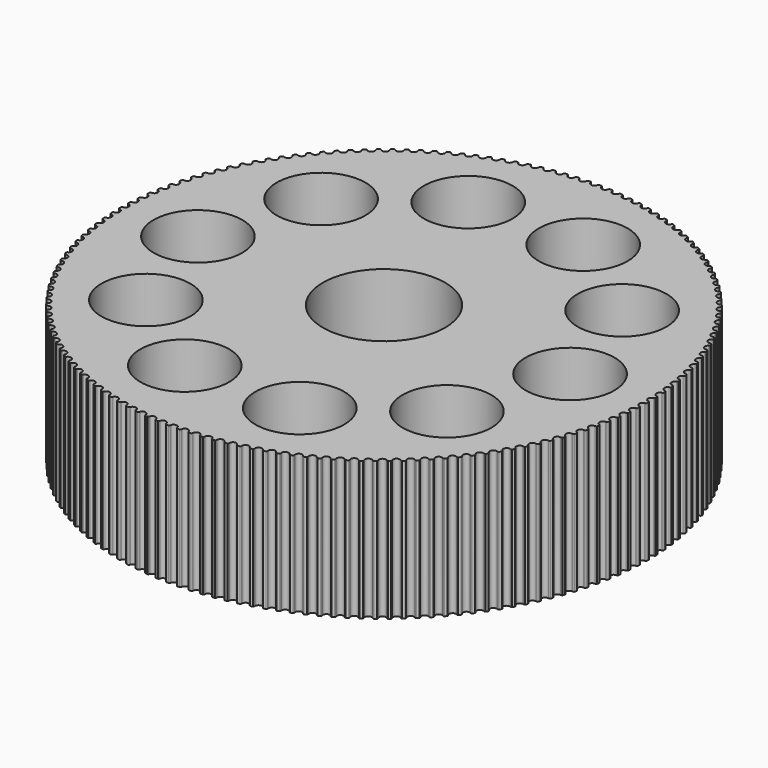
from build123d import *

# Parameters (mm, degrees)
F0_R     = 8
F0_R_2   = 11
F1_DEPTH = 25


# Not quite as in the source:
# - ends of sketch curves that miss each other by under 0.0002 mm in the source are joined


with BuildPart() as f1:
    # F0 (on Top) → F1 (new body)
    with BuildSketch(Plane.XY):
        with BuildLine():
            ThreePointArc((5.182516975, 47.241582772), (4.967715793, 47.2646530168), (4.7528119592, 47.2867465944))
            ThreePointArc((4.7528119592, 47.2867465944), (4.6733752274, 47.2476348408), (4.6144722817, 47.181525833))
            ThreePointArc((4.6144722817, 47.181525833), (4.5794914549, 47.1137403923), (4.5526895492, 47.0423248299))
            ThreePointArc((4.5526895492, 47.0423248299), (3.9140899665, 46.611650764), (3.3562563263, 47.1427920436))
            ThreePointArc((3.3562563263, 47.1427920436), (3.3417398463, 47.2176777416), (3.3185532394, 47.2903480922))
            ThreePointArc((3.3185532394, 47.2903480922), (3.2714996134, 47.3653531389), (3.1996987411, 47.4171644391))
            ThreePointArc((3.1996987411, 47.4171644391), (2.9841198433, 47.4312202432), (2.7684790129, 47.4442952203))
            ThreePointArc((2.7684790129, 47.4442952203), (2.6907501452, 47.4018909549), (2.6346674009, 47.3333737845))
            ThreePointArc((2.6346674009, 47.3333737845), (2.6025556228, 47.2641831956), (2.5787678102, 47.1917080502))
            ThreePointArc((2.5787678102, 47.1917080502), (1.9587633402, 46.7346701592), (1.3791768864, 47.2419849799))
            ThreePointArc((1.3791768864, 47.2419849799), (1.3615372148, 47.3161971817), (1.3353277912, 47.3878329094))
            ThreePointArc((1.3353277912, 47.3878329094), (1.2851750123, 47.460802605), (1.2112670238, 47.5095620579))
            ThreePointArc((1.2112670238, 47.5095620579), (0.9952887831, 47.5145769763), (0.7792900062, 47.5186103762))
            ThreePointArc((0.7792900062, 47.5186103762), (0.7034046202, 47.4729886965), (0.6502402175, 47.4021828946))
            ThreePointArc((0.6502402175, 47.4021828946), (0.6210538129, 47.3317080547), (0.6003217543, 47.2583000541))
            ThreePointArc((0.6003217543, 47.2583000541), (0, 46.7757), (-0.6003218986, 47.2583000223))
            ThreePointArc((-0.6003218986, 47.2583000223), (-0.6210538129, 47.3317080547), (-0.6502398609, 47.4021830674))
            ThreePointArc((-0.6502398609, 47.4021830674), (-0.7034037821, 47.4729888426), (-0.7792887875, 47.5186105849))
            ThreePointArc((-0.7792887875, 47.5186105849), (-0.9952877835, 47.5145769973), (-1.2112659942, 47.5095617712))
            ThreePointArc((-1.2112659942, 47.5095617712), (-1.2851745402, 47.4608030682), (-1.33532756, 47.387833243))
            ThreePointArc((-1.33532756, 47.387833243), (-1.3615362398, 47.3161970985), (-1.3791761881, 47.2419848567))
            ThreePointArc((-1.3791761881, 47.2419848567), (-1.9587632125, 46.7346701646), (-2.5787673524, 47.1917079068))
            ThreePointArc((-2.5787673524, 47.1917079068), (-2.6025555759, 47.2641830767), (-2.634667122, 47.3333739344))
            ThreePointArc((-2.634667122, 47.3333739344), (-2.6907496945, 47.4018914102), (-2.7684789183, 47.4442952581))
            ThreePointArc((-2.7684789183, 47.4442952581), (-2.9841193455, 47.4312202745), (-3.1996980149, 47.4171652212))
            ThreePointArc((-3.1996980149, 47.4171652212), (-3.2714993029, 47.3653534701), (-3.3185525607, 47.2903478308))
            ThreePointArc((-3.3185525607, 47.2903478308), (-3.3417389071, 47.2176775034), (-3.3562556365, 47.1427919514))
            ThreePointArc((-3.3562556365, 47.1427919514), (-3.9140899665, 46.611650764), (-4.5526894017, 47.0423248756))
            ThreePointArc((-4.5526894017, 47.0423248756), (-4.5794906183, 47.1137407605), (-4.6144714956, 47.181526299))
            ThreePointArc((-4.6144714956, 47.181526299), (-4.6733744303, 47.2476349951), (-4.7528110303, 47.2867468883))
            ThreePointArc((-4.7528110303, 47.2867468883), (-4.967714804, 47.2646531208), (-5.1825159869, 47.2415828804))
            ThreePointArc((-5.1825159869, 47.2415828804), (-5.252084897, 47.1868097785), (-5.2959557886, 47.1098989286))
            ThreePointArc((-5.2959557886, 47.1098989286), (-5.316079283, 47.0363217043), (-5.3274473912, 46.9608940357))
            ThreePointArc((-5.3274473912, 46.9608940357), (-5.8625494357, 46.4068599016), (-6.5186230792, 46.8104139718))
            ThreePointArc((-6.5186230792, 46.8104139718), (-6.5483919332, 46.8806448289), (-6.5861806975, 46.9469061969))
            ThreePointArc((-6.5861806975, 46.9469061969), (-6.6478009852, 47.0104901276), (-6.7288059192, 47.0462413564))
            ThreePointArc((-6.7288059192, 47.0462413564), (-6.9425957149, 47.0151676562), (-7.1562419661, 46.9831227775))
            ThreePointArc((-7.1562419661, 46.9831227775), (-7.2234562907, 46.9254845338), (-7.2640681919, 46.846804056))
            ThreePointArc((-7.2640681919, 46.846804056), (-7.2810926464, 46.7724485845), (-7.2892921509, 46.6966110074))
            ThreePointArc((-7.2892921509, 46.6966110074), (-7.8007249602, 46.1206548928), (-8.4731222646, 46.4963818931))
            ThreePointArc((-8.4731222646, 46.4963818931), (-8.5058058225, 46.5653043544), (-8.5463360323, 46.629924977))
            ThreePointArc((-8.5463360323, 46.629924977), (-8.6105643855, 46.6908725899), (-8.6929949517, 46.723200264))
            ThreePointArc((-8.6929949517, 46.723200264), (-8.9052965732, 46.6832016677), (-9.117414043, 46.64223822))
            ThreePointArc((-9.117414043, 46.64223822), (-9.1821560782, 46.5818362081), (-9.2194374834, 46.5015241193))
            ThreePointArc((-9.2194374834, 46.5015241193), (-9.2333329101, 46.426521141), (-9.2383494946, 46.3504070035))
            ThreePointArc((-9.2383494946, 46.3504070035), (-9.7252146618, 45.7535382711), (-10.4127566221, 46.1007787177))
            ThreePointArc((-10.4127566221, 46.1007787177), (-10.4482974147, 46.1682721976), (-10.4914981811, 46.2311388592))
            ThreePointArc((-10.4914981811, 46.2311388592), (-10.5582224722, 46.2893439391), (-10.6419349341, 46.3181914707))
            ThreePointArc((-10.6419349341, 46.3181914707), (-10.8523751931, 46.2693373377), (-11.0625910717, 46.2195272994))
            ThreePointArc((-11.0625910717, 46.2195272994), (-11.1247466028, 46.156466792), (-11.158632078, 46.0746640158))
            ThreePointArc((-11.158632078, 46.0746640158), (-11.1693742669, 45.9991451694), (-11.1711991686, 45.9228879941))
            ThreePointArc((-11.1711991686, 45.9228879941), (-11.6326433294, 45.306155295), (-12.334122955, 45.6243000227))
            ThreePointArc((-12.334122955, 45.6243000227), (-12.372459241, 45.6902458175), (-12.4182547156, 45.7512482408))
            ThreePointArc((-12.4182547156, 45.7512482408), (-12.4873576813, 45.806607327), (-12.5722040055, 45.8319239439))
            ThreePointArc((-12.5722040055, 45.8319239439), (-12.7804140886, 45.7743010949), (-12.9883599345, 45.7157317694))
            ThreePointArc((-12.9883599345, 45.7157317694), (-13.0478198358, 45.6501238029), (-13.0782501365, 45.5669740218))
            ThreePointArc((-13.0782501365, 45.5669740218), (-13.0858208354, 45.4910711783), (-13.0844507157, 45.4148040218))
            ThreePointArc((-13.0844507157, 45.4148040218), (-13.5196641554, 44.7792897847), (-14.2338505916, 45.0677802283))
            ThreePointArc((-14.2338505916, 45.0677802283), (-14.2749154334, 45.1320625096), (-14.3232252313, 45.1910937869))
            ThreePointArc((-14.3232252313, 45.1910937869), (-14.3945853729, 45.2435116639), (-14.4804180013, 45.2652529759))
            ThreePointArc((-14.4804180013, 45.2652529759), (-14.6860322599, 45.1989610662), (-14.8913430809, 45.1317352452))
            ThreePointArc((-14.8913430809, 45.1317352452), (-14.948003989, 45.0636951996), (-14.9749258079, 44.9793440943))
            ThreePointArc((-14.9749258079, 44.9793440943), (-14.9793115615, 44.9031908546), (-14.9747489747, 44.827048003))
            ThreePointArc((-14.9747489747, 44.827048003), (-15.3829670472, 44.1738658032), (-16.1086081109, 44.4321959318))
            ThreePointArc((-16.1086081109, 44.4321959318), (-16.1523281984, 44.4947027357), (-16.2030676277, 44.551659373))
            ThreePointArc((-16.2030676277, 44.551659373), (-16.2765610953, 44.60104224), (-16.3632289993, 44.6191700495))
            ThreePointArc((-16.3632289993, 44.6191700495), (-16.5658867493, 44.5443264761), (-16.7682020755, 44.4685622002))
            ThreePointArc((-16.7682020755, 44.4685622002), (-16.8219632166, 44.3982084522), (-16.8453288376, 44.3128039879))
            ThreePointArc((-16.8453288376, 44.3128039879), (-16.8465225529, 44.2365339418), (-16.8387753919, 44.1606489366))
            ThreePointArc((-16.8387753919, 44.1606489366), (-17.2192833212, 43.4909459416), (-17.9551052486, 43.7186628322))
            ThreePointArc((-17.9551052486, 43.7186628322), (-18.0014044539, 43.7792843025), (-18.0544846773, 43.8340663516))
            ThreePointArc((-18.0544846773, 43.8340663516), (-18.1299814951, 43.8803278162), (-18.2173319905, 43.8948106643))
            ThreePointArc((-18.2173319905, 43.8948106643), (-18.4166778941, 43.8115464272), (-18.6156432013, 43.7273764729))
            ThreePointArc((-18.6156432013, 43.7273764729), (-18.6664117427, 43.6548332953), (-18.6861804189, 43.5685249811))
            ThreePointArc((-18.6861804189, 43.5685249811), (-18.6841788985, 43.4922719475), (-18.6732608746, 43.4167780257))
            ThreePointArc((-18.6732608746, 43.4167780257), (-19.0253908784, 42.7317279858), (-19.7701033628, 42.9284317324))
            ThreePointArc((-19.7701033628, 42.9284317324), (-19.8189007922, 42.9870610958), (-19.8742285317, 43.0395723695))
            ThreePointArc((-19.8742285317, 43.0395723695), (-19.9515957027, 43.0826325416), (-20.0394759993, 43.0934449907))
            ThreePointArc((-20.0394759993, 43.0934449907), (-20.2351605671, 43.0019057929), (-20.4304268886, 42.909477766))
            ThreePointArc((-20.4304268886, 42.909477766), (-20.4781132708, 42.8348725168), (-20.4942506816, 42.7478119936))
            ThreePointArc((-20.4942506816, 42.7478119936), (-20.489056513, 42.671709629), (-20.4749866223, 42.5967390941))
            ThreePointArc((-20.4749866223, 42.5967390941), (-20.7981218958, 41.8975447723), (-21.550417902, 42.0628910788))
            ThreePointArc((-21.550417902, 42.0628910788), (-21.6016275113, 42.1194248834), (-21.6591051326, 42.1695728287))
            ThreePointArc((-21.6591051326, 42.1695728287), (-21.7382077113, 42.2093558082), (-21.8264639784, 42.2164788081))
            ThreePointArc((-21.8264639784, 42.2164788081), (-22.0181435968, 42.1168253498), (-22.2093682376, 42.0163014494))
            ThreePointArc((-22.2093682376, 42.0163014494), (-22.2538881422, 41.9397645577), (-22.2663654759, 41.8521050269))
            ThreePointArc((-22.2663654759, 41.8521050269), (-22.2579906662, 41.7762866169), (-22.2407936577, 41.7019708065))
            ThreePointArc((-22.2407936577, 41.7019708065), (-22.5343648664, 40.9898586918), (-23.2929249668, 41.123557029))
            ThreePointArc((-23.2929249668, 41.123557029), (-23.34645754, 41.1778967974), (-23.4059849904, 41.2255940135))
            ThreePointArc((-23.4059849904, 41.2255940135), (-23.4866846287, 41.2620289953), (-23.5751619171, 41.2654494664))
            ThreePointArc((-23.5751619171, 41.2654494664), (-23.7625000421, 41.1578572906), (-23.9493470717, 41.049414123))
            ThreePointArc((-23.9493470717, 41.049414123), (-23.9906227257, 40.9710801577), (-23.9994183098, 40.8829750645))
            ThreePointArc((-23.9994183098, 40.8829750645), (-23.9878753363, 40.8075742905), (-23.967581571, 40.734044146))
            ThreePointArc((-23.967581571, 40.734044146), (-24.2310758299, 40.0102618952), (-24.9945696971, 40.112077336))
            ThreePointArc((-24.9945696971, 40.112077336), (-25.0503298822, 40.164128868), (-25.1118026268, 40.2092915759))
            ThreePointArc((-25.1118026268, 40.2092915759), (-25.1939571522, 40.2423151203), (-25.2824999304, 40.2420276497))
            ThreePointArc((-25.2824999304, 40.2420276497), (-25.4651682323, 40.1266847858), (-25.6473102513, 40.010512392))
            ThreePointArc((-25.6473102513, 40.010512392), (-25.6852698626, 39.9305184783), (-25.6903684389, 39.8421220763))
            ThreePointArc((-25.6903684389, 39.8421220763), (-25.6756783405, 39.76727076), (-25.6523232271, 39.694654912))
            ThreePointArc((-25.6523232271, 39.694654912), (-25.8852770599, 38.9604741196), (-26.6523645845, 39.0302283945))
            ThreePointArc((-26.6523645845, 39.0302283945), (-26.7102561883, 39.0798986644), (-26.7735662519, 39.1224475731))
            ThreePointArc((-26.7735662519, 39.1224475731), (-26.8570310864, 39.1520020268), (-26.9454837989, 39.1480071706))
            ThreePointArc((-26.9454837989, 39.1480071706), (-27.1231622388, 39.0251162096), (-27.3002800877, 38.901418125))
            ThreePointArc((-27.3002800877, 38.901418125), (-27.334856433, 38.8199051815), (-27.3362486703, 38.731373059))
            ThreePointArc((-27.3362486703, 38.731373059), (-27.3184367896, 38.6572023087), (-27.2920612072, 38.5856279095))
            ThreePointArc((-27.2920612072, 38.5856279095), (-27.4940660954, 37.8423364816), (-28.2634016352, 37.879907411))
            ThreePointArc((-28.2634016352, 37.879907411), (-28.3233225159, 37.9271098296), (-28.3883588605, 37.9669702608))
            ThreePointArc((-28.3883588605, 37.9669702608), (-28.4729886807, 37.9930038603), (-28.5611971074, 37.9853083739))
            ThreePointArc((-28.5611971074, 37.9853083739), (-28.7335730098, 37.8550842964), (-28.9053551048, 37.7240781367))
            ThreePointArc((-28.9053551048, 37.7240781367), (-28.9364879218, 37.6411887841), (-28.9341720483, 37.5526759893))
            ThreePointArc((-28.9341720483, 37.5526759893), (-28.9132696795, 37.4793161686), (-28.8839200196, 37.4089089904))
            ThreePointArc((-28.8839200196, 37.4089089904), (-29.0546218419, 36.6578103378), (-29.8248559799, 36.6631320247))
            ThreePointArc((-29.8248559799, 36.6631320247), (-29.8867007266, 36.7077838547), (-29.9533490818, 36.7448858304))
            ThreePointArc((-29.9533490818, 36.7448858304), (-30.0389945211, 36.7673524992), (-30.1268029854, 36.7559699561))
            ThreePointArc((-30.1268029854, 36.7559699561), (-30.2935747545, 36.6186421593), (-30.4597202933, 36.4805573512))
            ThreePointArc((-30.4597202933, 36.4805573512), (-30.4873548316, 36.3964365062), (-30.4813341671, 36.3080979554))
            ThreePointArc((-30.4813341671, 36.3080979554), (-30.4573782075, 36.2356780829), (-30.4251059659, 36.1665620185))
            ThreePointArc((-30.4251059659, 36.1665620185), (-30.5642054256, 35.4089732771), (-31.3339872568, 35.3820366566))
            ThreePointArc((-31.3339872568, 35.3820366566), (-31.3976474883, 35.4240595475), (-31.465791003, 35.458337993))
            ThreePointArc((-31.465791003, 35.458337993), (-31.5523022038, 35.4771984151), (-31.6395570306, 35.4621490804))
            ThreePointArc((-31.6395570306, 35.4621490804), (-31.8004317506, 35.3179581159), (-31.9606490615, 35.1730370677))
            ThreePointArc((-31.9606490615, 35.1730370677), (-31.9847373336, 35.0878329951), (-31.9750225325, 34.9998238337))
            ThreePointArc((-31.9750225325, 34.9998238337), (-31.9480542684, 34.9284709196), (-31.9129161576, 34.8607669061))
            ThreePointArc((-31.9129161576, 34.8607669061), (-32.0201694485, 34.0980176922), (-32.7881478533, 34.0388692144))
            ThreePointArc((-32.7881478533, 34.0388692144), (-32.8535122402, 34.0781896993), (-32.9230317324, 34.1095846992))
            ThreePointArc((-32.9230317324, 34.1095846992), (-33.010256823, 34.1248059667), (-33.0968049253, 34.106115826))
            ThreePointArc((-33.0968049253, 34.106115826), (-33.2515000415, 33.9553143114), (-33.4055081637, 33.8038111657))
            ThreePointArc((-33.4055081637, 33.8038111657), (-33.4260067003, 33.7176729901), (-33.4126149432, 33.6301480204))
            ThreePointArc((-33.4126149432, 33.6301480204), (-33.3826833245, 33.5599869553), (-33.3447409964, 33.4938140023))
            ThreePointArc((-33.3447409964, 33.4938140023), (-33.419959633, 32.7272432445), (-34.1847867953, 32.6359863276))
            ThreePointArc((-34.1847867953, 32.6359863276), (-34.2517405999, 32.6725350168), (-34.3225139108, 32.7009912658))
            ThreePointArc((-34.3225139108, 32.7009912658), (-34.4102997305, 32.7125460471), (-34.4959889429, 32.6902478811))
            ThreePointArc((-34.4959889429, 32.6902478811), (-34.6442340207, 32.5331012066), (-34.7917627518, 32.375281769))
            ThreePointArc((-34.7917627518, 32.375281769), (-34.8086358877, 32.2883611476), (-34.7915910147, 32.201473994))
            ThreePointArc((-34.7915910147, 32.201473994), (-34.7587472343, 32.1326275223), (-34.718066857, 32.0681011024))
            ThreePointArc((-34.718066857, 32.0681011024), (-34.7611189856, 31.2990525246), (-35.5214547493, 31.1758494415))
            ThreePointArc((-35.5214547493, 31.1758494415), (-35.5898799994, 31.2095613052), (-35.6617820776, 31.235028732))
            ThreePointArc((-35.6617820776, 31.235028732), (-35.7499752272, 31.2428984823), (-35.8346562444, 31.2170314592))
            ThreePointArc((-35.8346562444, 31.2170314592), (-35.9761900627, 31.053814155), (-36.1169804859, 30.8899554156))
            ThreePointArc((-36.1169804859, 30.8899554156), (-36.1301995967, 30.8024042), (-36.1095311663, 30.7163069241))
            ThreePointArc((-36.1095311663, 30.7163069241), (-36.0738325389, 30.6488964912), (-36.0304858127, 30.5861301463))
            ThreePointArc((-36.0304858127, 30.5861301463), (-36.0412958654, 29.8159532879), (-36.7958050105, 29.6610179795))
            ThreePointArc((-36.7958050105, 29.6610179795), (-36.8655820838, 29.6918356831), (-36.9384880184, 29.7142699246))
            ThreePointArc((-36.9384880184, 29.7142699246), (-37.0269330204, 29.7184396086), (-37.1104562934, 29.6890494996))
            ThreePointArc((-37.1104562934, 29.6890494996), (-37.2450315898, 29.5200482194), (-37.3788371443, 29.3504371133))
            ThreePointArc((-37.3788371443, 29.3504371133), (-37.388378177, 29.2624096081), (-37.3641226412, 29.1772536741))
            ThreePointArc((-37.3641226412, 29.1772536741), (-37.325632506, 29.1113970272), (-37.279695289, 29.0505007541))
            ThreePointArc((-37.279695289, 29.0505007541), (-37.2582441495, 28.280546806), (-38.0056038208, 28.0941523881))
            ThreePointArc((-38.0056038208, 28.0941523881), (-38.0766100533, 28.1220203219), (-38.1503910405, 28.1413817982))
            ThreePointArc((-38.1503910405, 28.1413817982), (-38.2389330674, 28.1418445383), (-38.3211524303, 28.1089826669))
            ThreePointArc((-38.3211524303, 28.1089826669), (-38.4485325141, 27.9344943129), (-38.5751179819, 27.759428987))
            ThreePointArc((-38.5751179819, 27.759428987), (-38.5809647654, 27.6710787667), (-38.5531644362, 27.5870127548))
            ThreePointArc((-38.5531644362, 27.5870127548), (-38.5119502655, 27.5228262248), (-38.4635036298, 27.4639073427))
            ThreePointArc((-38.4635036298, 27.4639073427), (-38.4098288032, 26.6955270733), (-39.1487269601, 26.4779990969))
            ThreePointArc((-39.1487269601, 26.4779990969), (-39.2208382091, 26.5028702875), (-39.2953659494, 26.5191253217))
            ThreePointArc((-39.2953659494, 26.5191253217), (-39.3838493162, 26.5158789126), (-39.4646199653, 26.4796029509))
            ThreePointArc((-39.4646199653, 26.4796029509), (-39.584581656, 26.2999338425), (-39.7037251846, 26.1197211215))
            ThreePointArc((-39.7037251846, 26.1197211215), (-39.7058670803, 26.0312038152), (-39.6745710203, 25.9483759874))
            ThreePointArc((-39.6745710203, 25.9483759874), (-39.6307057529, 25.8859707396), (-39.5798340393, 25.8291319605))
            ThreePointArc((-39.5798340393, 25.8291319605), (-39.4940294685, 25.0636730523), (-40.2231711419, 24.8153946099))
            ThreePointArc((-40.2231711419, 24.8153946099), (-40.2962602989, 24.8372241426), (-40.3714030081, 24.8503439297))
            ThreePointArc((-40.3714030081, 24.8503439297), (-40.4596729799, 24.8433954665), (-40.5388538436, 24.8037687972))
            ThreePointArc((-40.5388538436, 24.8037687972), (-40.6511863672, 24.6192337806), (-40.7626788627, 24.4341899177))
            ThreePointArc((-40.7626788627, 24.4341899177), (-40.7611115635, 24.345660489), (-40.7263742918, 24.2642158021))
            ThreePointArc((-40.7263742918, 24.2642158021), (-40.67993449, 24.2037021826), (-40.6267272675, 24.1490437072))
            ThreePointArc((-40.6267272675, 24.1490437072), (-40.5089445102, 23.3878499906), (-41.2270490314, 23.1092559009))
            ThreePointArc((-41.2270490314, 23.1092559009), (-41.3009880302, 23.1280054435), (-41.3766139898, 23.1379671412))
            ThreePointArc((-41.3766139898, 23.1379671412), (-41.464515834, 23.127328707), (-41.5419682039, 23.0844212428))
            ThreePointArc((-41.5419682039, 23.0844212428), (-41.6464748459, 22.8953435858), (-41.7501208681, 22.7057929283))
            ThreePointArc((-41.7501208681, 22.7057929283), (-41.7448474212, 22.6174066983), (-41.706729842, 22.5374881171))
            ThreePointArc((-41.706729842, 22.5374881171), (-41.6577969362, 22.4789725176), (-41.6023477515, 22.4265902961))
            ThreePointArc((-41.6023477515, 22.4265902961), (-41.4527923686, 21.6709962225), (-42.1586011383, 21.3625754906))
            ThreePointArc((-42.1586011383, 21.3625754906), (-42.2332607783, 21.3782126624), (-42.3092379781, 21.3849987192))
            ThreePointArc((-42.3092379781, 21.3849987192), (-42.3966168796, 21.3706874774), (-42.4722040722, 21.324574079))
            ThreePointArc((-42.4722040722, 21.324574079), (-42.5687013144, 21.1312870741), (-42.6643184743, 20.9375632328))
            ThreePointArc((-42.6643184743, 20.9375632328), (-42.6553489686, 20.8494754388), (-42.6139186703, 20.7712232664))
            ThreePointArc((-42.6139186703, 20.7712232664), (-42.5625776857, 20.7148076733), (-42.5049831261, 20.6647928363))
            ThreePointArc((-42.5049831261, 20.6647928363), (-42.3239189918, 19.9161238057), (-43.0161930939, 19.5784175862))
            ThreePointArc((-43.0161930939, 19.5784175862), (-43.0914416661, 19.59091457), (-43.1676360004, 19.5945130332))
            ThreePointArc((-43.1676360004, 19.5945130332), (-43.2543389388, 19.5765557765), (-43.3279289271, 19.5273179267))
            ThreePointArc((-43.3279289271, 19.5273179267), (-43.4162477291, 19.3301592886), (-43.5036688797, 19.1326009471))
            ThreePointArc((-43.5036688797, 19.1326009471), (-43.4910181921, 19.0449658422), (-43.446347061, 18.9685169463))
            ThreePointArc((-43.446347061, 18.9685169463), (-43.3926887641, 18.914301323), (-43.3330506322, 18.8667425212))
            ThreePointArc((-43.3330506322, 18.8667425212), (-43.1207941695, 18.1263128918), (-43.7983189585, 17.7599132265))
            ThreePointArc((-43.7983189585, 17.7599132265), (-43.8740253637, 17.7692480398), (-43.9503040358, 17.7696526705))
            ThreePointArc((-43.9503040358, 17.7696526705), (-44.0361790654, 17.7480803308), (-44.1076425287, 17.695803564))
            ThreePointArc((-44.1076425287, 17.695803564), (-44.1876275362, 17.4951192542), (-44.2666992324, 17.2940730908))
            ThreePointArc((-44.2666992324, 17.2940730908), (-44.2503896234, 17.2070450542), (-44.2025567121, 17.1325342755))
            ThreePointArc((-44.2025567121, 17.1325342755), (-44.1466751119, 17.0806131833), (-44.0850976956, 17.0355934722))
            ThreePointArc((-44.0850976956, 17.0355934722), (-43.8420205774, 16.304701544), (-44.503608888, 15.9102517981))
            ThreePointArc((-44.503608888, 15.9102517981), (-44.5796395493, 15.9164081413), (-44.6558680186, 15.9136181946))
            ThreePointArc((-44.6558680186, 15.9136181946), (-44.7407643979, 15.8884684921), (-44.8099761968, 15.8332451673))
            ThreePointArc((-44.8099761968, 15.8332451673), (-44.8814869352, 15.6293875596), (-44.9520701664, 15.4252070571))
            ThreePointArc((-44.9520701664, 15.4252070571), (-44.9321311842, 15.3389379316), (-44.8812197411, 15.2664952694))
            ThreePointArc((-44.8812197411, 15.2664952694), (-44.8232130285, 15.2169593728), (-44.7598042574, 15.1745575614))
            ThreePointArc((-44.7598042574, 15.1745575614), (-44.486333694, 14.4544860846), (-45.130823993, 14.0326780718))
            ThreePointArc((-45.130823993, 14.0326780718), (-45.2070455279, 14.0356447694), (-45.2830900296, 14.0296652142))
            ThreePointArc((-45.2830900296, 14.0296652142), (-45.3668588593, 14.0009828017), (-45.4336974285, 13.9429095539))
            ThreePointArc((-45.4336974285, 13.9429095539), (-45.4966090409, 13.7362364124), (-45.5585802332, 13.5292790693))
            ThreePointArc((-45.5585802332, 13.5292790693), (-45.5350457363, 13.4439206514), (-45.481145628, 13.3736734211))
            ThreePointArc((-45.481145628, 13.3736734211), (-45.4211154877, 13.3266103507), (-45.3559869186, 13.286901153))
            ThreePointArc((-45.3559869186, 13.286901153), (-45.0526032262, 12.5789123906), (-45.678864028, 12.1304854988))
            ThreePointArc((-45.678864028, 12.1304854988), (-45.7551427565, 12.1302589071), (-45.8308700452, 12.12110025))
            ThreePointArc((-45.8308700452, 12.12110025), (-45.9133644537, 12.0889350205), (-45.977712727, 12.0281138048))
            ThreePointArc((-45.977712727, 12.0281138048), (-46.0319146701, 11.8189871313), (-46.0851650842, 11.6096160212))
            ThreePointArc((-46.0851650842, 11.6096160212), (-46.058076808, 11.525318112), (-46.0012822224, 11.4573897259))
            ThreePointArc((-46.0012822224, 11.4573897259), (-45.9393341101, 11.4128819023), (-45.8726000229, 11.3759349522))
            ThreePointArc((-45.8726000229, 11.3759349522), (-45.5398345238, 10.6812722711), (-46.1467679905, 10.2070136901))
            ThreePointArc((-46.1467679905, 10.2070136901), (-46.2229704614, 10.2035914228), (-46.2982479096, 10.1912695974))
            ThreePointArc((-46.2982479096, 10.1912695974), (-46.3793228466, 10.155678182), (-46.4410675344, 10.0922156956))
            ThreePointArc((-46.4410675344, 10.0922156956), (-46.4864647311, 9.8810030768), (-46.5309008323, 9.6695859651))
            ThreePointArc((-46.5309008323, 9.6695859651), (-46.5003066861, 9.5864962678), (-46.4407171363, 9.5210058169))
            ThreePointArc((-46.4407171363, 9.5210058169), (-46.3769588873, 9.4791314955), (-46.3087358569, 9.4450113338))
            ThreePointArc((-46.3087358569, 9.4450113338), (-45.9471736584, 8.7648925287), (-46.5337140042, 8.2656341504))
            ThreePointArc((-46.5337140042, 8.2656341504), (-46.6097069416, 8.2590243188), (-46.6844029572, 8.243560841))
            ThreePointArc((-46.6844029572, 8.243560841), (-46.7639164208, 8.2046056402), (-46.8229495371, 8.1386133198))
            ThreePointArc((-46.8229495371, 8.1386133198), (-46.8594616969, 7.9256844802), (-46.8950055782, 7.7125920951))
            ThreePointArc((-46.8950055782, 7.7125920951), (-46.8609583651, 7.6308565586), (-46.7986790106, 7.5679189844))
            ThreePointArc((-46.7986790106, 7.5679189844), (-46.7332236904, 7.528750774), (-46.6636318399, 7.4975174212))
            ThreePointArc((-46.6636318399, 7.4975174212), (-46.273906035, 6.8331360048), (-46.8390249697, 6.309753568))
            ThreePointArc((-46.8390249697, 6.309753568), (-46.9146742065, 6.2999674873), (-46.9886569005, 6.2813896837))
            ThreePointArc((-46.9886569005, 6.2813896837), (-47.066469496, 6.2391396243), (-47.1226873331, 6.1707331799))
            ThreePointArc((-47.1226873331, 6.1707331799), (-47.1502511572, 5.9564621055), (-47.1768404981, 5.7420680606))
            ThreePointArc((-47.1768404981, 5.7420680606), (-47.1394001075, 5.661829962), (-47.0745396223, 5.6015556078))
            ThreePointArc((-47.0745396223, 5.6015556078), (-47.0075019852, 5.5651619982), (-46.9366632199, 5.5368703393))
            ThreePointArc((-46.9366632199, 5.5368703393), (-46.5194573164, 4.8893921112), (-47.0621650589, 4.3428045248))
            ThreePointArc((-47.0621650589, 4.3428045248), (-47.1373377102, 4.3298589257), (-47.2104771775, 4.3081994915))
            ThreePointArc((-47.2104771775, 4.3081994915), (-47.2864523858, 4.2627279285), (-47.3397564144, 4.1920272019))
            ThreePointArc((-47.3397564144, 4.1920272019), (-47.3583231265, 3.9767896154), (-47.375911266, 3.7614700211))
            ThreePointArc((-47.375911266, 3.7614700211), (-47.335143999, 3.6828700419), (-47.2678161821, 3.6253646777))
            ThreePointArc((-47.2678161821, 3.6253646777), (-47.1993133329, 3.591810691), (-47.1273522197, 3.5665102343))
            ThreePointArc((-47.1273522197, 3.5665102343), (-46.68339893, 2.9370709332), (-47.2027410539, 2.3682363481))
            ThreePointArc((-47.2027410539, 2.3682363481), (-47.2773057718, 2.3521545361), (-47.3494741456, 2.3274513558))
            ThreePointArc((-47.3494741456, 2.3274513558), (-47.423478545, 2.2788373269), (-47.4737751834, 2.20596608))
            ThreePointArc((-47.4737751834, 2.20596608), (-47.4833125157, 1.990140079), (-47.4918685697, 1.7742730213))
            ThreePointArc((-47.4918685697, 1.7742730213), (-47.4478459212, 1.6974490126), (-47.3781693192, 1.6428133751))
            ThreePointArc((-47.3781693192, 1.6428133751), (-47.3083207728, 1.6121580297), (-47.2353629662, 1.5898931395))
            ThreePointArc((-47.2353629662, 1.5898931395), (-46.7654408053, 0.9795963131), (-47.2605069473, 0.3895127343))
            ThreePointArc((-47.2605069473, 0.3895127343), (-47.3343332695, 0.3703231254), (-47.4054041957, 0.3426194264))
            ThreePointArc((-47.4054041957, 0.3426194264), (-47.4773077897, 0.2909491973), (-47.5245087895, 0.2160359185))
            ThreePointArc((-47.5245087895, 0.2160359185), (-47.525, 0), (-47.5245089764, -0.2160359999))
            ThreePointArc((-47.5245089764, -0.2160359999), (-47.4773077897, -0.2909491973), (-47.4054041258, -0.3426192741))
            ThreePointArc((-47.4054041258, -0.3426192741), (-47.3343332695, -0.3703231254), (-47.2605070465, -0.3895132348))
            ThreePointArc((-47.2605070465, -0.3895132348), (-46.7654408053, -0.9795963131), (-47.2353629513, -1.5898932012))
            ThreePointArc((-47.2353629513, -1.5898932012), (-47.3083207728, -1.6121580297), (-47.3781691783, -1.6428136509))
            ThreePointArc((-47.3781691783, -1.6428136509), (-47.4478459212, -1.6974490126), (-47.4918683711, -1.7742728739))
            ThreePointArc((-47.4918683711, -1.7742728739), (-47.4833125157, -1.990140079), (-47.4737752759, -2.2059660128))
            ThreePointArc((-47.4737752759, -2.2059660128), (-47.423478545, -2.2788373269), (-47.3494740957, -2.3274512337))
            ThreePointArc((-47.3494740957, -2.3274512337), (-47.2773057718, -2.3521545361), (-47.2027410451, -2.3682362908))
            ThreePointArc((-47.2027410451, -2.3682362908), (-46.68339893, -2.9370709332), (-47.1273520283, -3.5665109014))
            ThreePointArc((-47.1273520283, -3.5665109014), (-47.1993133329, -3.591810691), (-47.267816432, -3.6253642351))
            ThreePointArc((-47.267816432, -3.6253642351), (-47.335143999, -3.6828700419), (-47.375911002, -3.7614699994))
            ThreePointArc((-47.375911002, -3.7614699994), (-47.3583231265, -3.9767896154), (-47.3397563824, -4.1920270339))
            ThreePointArc((-47.3397563824, -4.1920270339), (-47.2864523858, -4.2627279285), (-47.2104773469, -4.3081999604))
            ThreePointArc((-47.2104773469, -4.3081999604), (-47.1373377102, -4.3298589257), (-47.0621650182, -4.3428041617))
            ThreePointArc((-47.0621650182, -4.3428041617), (-46.5194573164, -4.8893921112), (-46.936662938, -5.5368711863))
            ThreePointArc((-46.936662938, -5.5368711863), (-47.0075019852, -5.5651619982), (-47.0745401551, -5.6015547504))
            ThreePointArc((-47.0745401551, -5.6015547504), (-47.1394001075, -5.661829962), (-47.1768397715, -5.7420680569))
            ThreePointArc((-47.1768397715, -5.7420680569), (-47.1502511572, -5.9564621055), (-47.1226875126, -6.1707330671))
            ThreePointArc((-47.1226875126, -6.1707330671), (-47.066469496, -6.2391396243), (-46.9886570713, -6.2813902266))
            ThreePointArc((-46.9886570713, -6.2813902266), (-46.9146742065, -6.2999674873), (-46.8390249651, -6.309753502))
            ThreePointArc((-46.8390249651, -6.309753502), (-46.273906035, -6.8331360048), (-46.6636319445, -7.4975171462))
            ThreePointArc((-46.6636319445, -7.4975171462), (-46.7332236904, -7.528750774), (-46.7986790305, -7.5679189552))
            ThreePointArc((-46.7986790305, -7.5679189552), (-46.8609583651, -7.6308565586), (-46.8950050149, -7.712591997))
            ThreePointArc((-46.8950050149, -7.712591997), (-46.8594616969, -7.9256844802), (-46.8229495222, -8.1386130908))
            ThreePointArc((-46.8229495222, -8.1386130908), (-46.7639164208, -8.2046056402), (-46.6844029313, -8.2435607445))
            ThreePointArc((-46.6844029313, -8.2435607445), (-46.6097069416, -8.2590243188), (-46.5337139964, -8.2656338704))
            ThreePointArc((-46.5337139964, -8.2656338704), (-45.9471736584, -8.7648925287), (-46.3087359821, -9.4450110417))
            ThreePointArc((-46.3087359821, -9.4450110417), (-46.3769588873, -9.4791314955), (-46.4407167504, -9.5210063354))
            ThreePointArc((-46.4407167504, -9.5210063354), (-46.5003066861, -9.5864962678), (-46.5309009411, -9.6695860095))
            ThreePointArc((-46.5309009411, -9.6695860095), (-46.4864647311, -9.8810030768), (-46.4410680435, -10.0922160094))
            ThreePointArc((-46.4410680435, -10.0922160094), (-46.3793228466, -10.155678182), (-46.2982479055, -10.1912695794))
            ThreePointArc((-46.2982479055, -10.1912695794), (-46.2229704614, -10.2035914228), (-46.1467680011, -10.2070129198))
            ThreePointArc((-46.1467680011, -10.2070129198), (-45.5398345238, -10.6812722711), (-45.8725998811, -11.375935248))
            ThreePointArc((-45.8725998811, -11.375935248), (-45.9393341101, -11.4128819023), (-46.0012822591, -11.4573896807))
            ThreePointArc((-46.0012822591, -11.4573896807), (-46.058076808, -11.525318112), (-46.0851646054, -11.6096160469))
            ThreePointArc((-46.0851646054, -11.6096160469), (-46.0319146701, -11.8189871313), (-45.97771306, -12.0281140157))
            ThreePointArc((-45.97771306, -12.0281140157), (-45.9133644537, -12.0889350205), (-45.8308699987, -12.1210999929))
            ThreePointArc((-45.8308699987, -12.1210999929), (-45.7551427565, -12.1302589071), (-45.6788639813, -12.1304863352))
            ThreePointArc((-45.6788639813, -12.1304863352), (-45.0526032262, -12.5789123906), (-45.3559871538, -13.2869007108))
            ThreePointArc((-45.3559871538, -13.2869007108), (-45.4211154877, -13.3266103507), (-45.4811456697, -13.3736733739))
            ThreePointArc((-45.4811456697, -13.3736733739), (-45.5350457363, -13.4439206514), (-45.558579583, -13.5292790319))
            ThreePointArc((-45.558579583, -13.5292790319), (-45.4966090409, -13.7362364124), (-45.4336977161, -13.9429099129))
            ThreePointArc((-45.4336977161, -13.9429099129), (-45.3668588593, -14.0009828017), (-45.2830900248, -14.0296651796))
            ThreePointArc((-45.2830900248, -14.0296651796), (-45.2070455279, -14.0356447694), (-45.1308240188, -14.0326778082))
            ThreePointArc((-45.1308240188, -14.0326778082), (-44.486333694, -14.4544860846), (-44.7598039089, -15.1745581551))
            ThreePointArc((-44.7598039089, -15.1745581551), (-44.8232130285, -15.2169593728), (-44.8812199026, -15.2664951013))
            ThreePointArc((-44.8812199026, -15.2664951013), (-44.9321311842, -15.3389379316), (-44.9520701714, -15.4252069941))
            ThreePointArc((-44.9520701714, -15.4252069941), (-44.8814869352, -15.6293875596), (-44.8099762842, -15.8332451004))
            ThreePointArc((-44.8099762842, -15.8332451004), (-44.7407643979, -15.8884684921), (-44.6558679792, -15.9136177825))
            ThreePointArc((-44.6558679792, -15.9136177825), (-44.5796395493, -15.9164081413), (-44.5036088677, -15.9102519423))
            ThreePointArc((-44.5036088677, -15.9102519423), (-43.8420205774, -16.304701544), (-44.0850975841, -17.0355936451))
            ThreePointArc((-44.0850975841, -17.0355936451), (-44.1466751119, -17.0806131833), (-44.2025566728, -17.1325343131))
            ThreePointArc((-44.2025566728, -17.1325343131), (-44.2503896234, -17.2070450542), (-44.2666985407, -17.2940729966))
            ThreePointArc((-44.2666985407, -17.2940729966), (-44.1876275362, -17.4951192542), (-44.1076427537, -17.6958039012))
            ThreePointArc((-44.1076427537, -17.6958039012), (-44.0361790654, -17.7480803308), (-43.9503040365, -17.7696526825))
            ThreePointArc((-43.9503040365, -17.7696526825), (-43.8740253637, -17.7692480398), (-43.7983189381, -17.7599133378))
            ThreePointArc((-43.7983189381, -17.7599133378), (-43.1207941695, -18.1263128918), (-43.3330508041, -18.8667422777))
            ThreePointArc((-43.3330508041, -18.8667422777), (-43.3926887641, -18.914301323), (-43.4463470408, -18.9685169641))
            ThreePointArc((-43.4463470408, -18.9685169641), (-43.4910181921, -19.0449658422), (-43.5036684056, -19.1326009706))
            ThreePointArc((-43.5036684056, -19.1326009706), (-43.4162477291, -19.3301592886), (-43.3279294345, -19.5273181958))
            ThreePointArc((-43.3279294345, -19.5273181958), (-43.2543389388, -19.5765557765), (-43.1676359969, -19.5945127282))
            ThreePointArc((-43.1676359969, -19.5945127282), (-43.0914416661, -19.59091457), (-43.0161930126, -19.5784179446))
            ThreePointArc((-43.0161930126, -19.5784179446), (-42.3239189918, -19.9161238057), (-42.5049835149, -20.6647923316))
            ThreePointArc((-42.5049835149, -20.6647923316), (-42.5625776857, -20.7148076733), (-42.6139187907, -20.7712231691))
            ThreePointArc((-42.6139187907, -20.7712231691), (-42.6553489686, -20.8494754388), (-42.6643182972, -20.9375630272))
            ThreePointArc((-42.6643182972, -20.9375630272), (-42.5687013144, -21.1312870741), (-42.4722045275, -21.3245742648))
            ThreePointArc((-42.4722045275, -21.3245742648), (-42.3966168796, -21.3706874774), (-42.3092379915, -21.384998281))
            ThreePointArc((-42.3092379915, -21.384998281), (-42.2332607783, -21.3782126624), (-42.1586010654, -21.3625757592))
            ThreePointArc((-42.1586010654, -21.3625757592), (-41.4527923686, -21.6709962225), (-41.6023476511, -22.4265904157))
            ThreePointArc((-41.6023476511, -22.4265904157), (-41.6577969362, -22.4789725176), (-41.7067302515, -22.5374878136))
            ThreePointArc((-41.7067302515, -22.5374878136), (-41.7448474212, -22.6174066983), (-41.7501204299, -22.7057929236))
            ThreePointArc((-41.7501204299, -22.7057929236), (-41.6464748459, -22.8953435858), (-41.5419682463, -23.0844211369))
            ThreePointArc((-41.5419682463, -23.0844211369), (-41.464515834, -23.127328707), (-41.3766139694, -23.137967423))
            ThreePointArc((-41.3766139694, -23.137967423), (-41.3009880302, -23.1280054435), (-41.2270490217, -23.1092559314))
            ThreePointArc((-41.2270490217, -23.1092559314), (-40.5089445102, -23.3878499906), (-40.6267271849, -24.1490437976))
            ThreePointArc((-40.6267271849, -24.1490437976), (-40.67993449, -24.2037021826), (-40.7263746743, -24.2642155428))
            ThreePointArc((-40.7263746743, -24.2642155428), (-40.7611115635, -24.345660489), (-40.7626785318, -24.4341899172))
            ThreePointArc((-40.7626785318, -24.4341899172), (-40.6511863672, -24.6192337806), (-40.5388538632, -24.8037689163))
            ThreePointArc((-40.5388538632, -24.8037689163), (-40.4596729799, -24.8433954665), (-40.3714029643, -24.8503443112))
            ThreePointArc((-40.3714029643, -24.8503443112), (-40.2962602989, -24.8372241426), (-40.2231710589, -24.8153948381))
            ThreePointArc((-40.2231710589, -24.8153948381), (-39.4940294685, -25.0636730523), (-39.579834039, -25.8291319608))
            ThreePointArc((-39.579834039, -25.8291319608), (-39.6307057529, -25.8859707396), (-39.6745711549, -25.9483759042))
            ThreePointArc((-39.6745711549, -25.9483759042), (-39.7058670803, -26.0312038152), (-39.703725343, -26.1197210756))
            ThreePointArc((-39.703725343, -26.1197210756), (-39.584581656, -26.2999338425), (-39.4646201592, -26.4796031068))
            ThreePointArc((-39.4646201592, -26.4796031068), (-39.3838493162, -26.5158789126), (-39.2953659596, -26.519125257))
            ThreePointArc((-39.2953659596, -26.519125257), (-39.2208382091, -26.5028702875), (-39.1487268819, -26.4779992867))
            ThreePointArc((-39.1487268819, -26.4779992867), (-38.4098288032, -26.6955270733), (-38.4635038722, -27.4639071183))
            ThreePointArc((-38.4635038722, -27.4639071183), (-38.5119502655, -27.5228262248), (-38.5531637227, -27.5870131559))
            ThreePointArc((-38.5531637227, -27.5870131559), (-38.5809647654, -27.6710787667), (-38.5751181217, -27.7594290322))
            ThreePointArc((-38.5751181217, -27.7594290322), (-38.4485325141, -27.9344943129), (-38.3211525541, -28.1089824064))
            ThreePointArc((-38.3211525541, -28.1089824064), (-38.2389330674, -28.1418445383), (-38.1503909155, -28.1413824214))
            ThreePointArc((-38.1503909155, -28.1413824214), (-38.0766100533, -28.1220203219), (-38.0056041002, -28.0941517831))
            ThreePointArc((-38.0056041002, -28.0941517831), (-37.2582441495, -28.280546806), (-37.2796951914, -29.0505008371))
            ThreePointArc((-37.2796951914, -29.0505008371), (-37.325632506, -29.1113970272), (-37.3641221959, -29.1772539004))
            ThreePointArc((-37.3641221959, -29.1772539004), (-37.388378177, -29.2624096081), (-37.3788372346, -29.3504370728))
            ThreePointArc((-37.3788372346, -29.3504370728), (-37.2450315898, -29.5200482194), (-37.1104564103, -29.6890493283))
            ThreePointArc((-37.1104564103, -29.6890493283), (-37.0269330204, -29.7184396086), (-36.9384879414, -29.7142702395))
            ThreePointArc((-36.9384879414, -29.7142702395), (-36.8655820838, -29.6918356831), (-36.7958050268, -29.6610179479))
            ThreePointArc((-36.7958050268, -29.6610179479), (-36.0412958654, -29.8159532879), (-36.0304860172, -30.5861299865))
            ThreePointArc((-36.0304860172, -30.5861299865), (-36.0738325389, -30.6488964912), (-36.1095305836, -30.7163071901))
            ThreePointArc((-36.1095305836, -30.7163071901), (-36.1301995967, -30.8024042), (-36.1169806838, -30.8899552439))
            ThreePointArc((-36.1169806838, -30.8899552439), (-35.9761900627, -31.053814155), (-35.8346562372, -31.2170312067))
            ThreePointArc((-35.8346562372, -31.2170312067), (-35.7499752272, -31.2428984823), (-35.6617819713, -31.2350290992))
            ThreePointArc((-35.6617819713, -31.2350290992), (-35.5898799994, -31.2095613052), (-35.5214550769, -31.1758488646))
            ThreePointArc((-35.5214550769, -31.1758488646), (-34.7611189856, -31.2990525246), (-34.7180666274, -32.0681012667))
            ThreePointArc((-34.7180666274, -32.0681012667), (-34.7587472343, -32.1326275223), (-34.7915911589, -32.2014739354))
            ThreePointArc((-34.7915911589, -32.2014739354), (-34.8086358877, -32.2883611476), (-34.7917623504, -32.3752817372))
            ThreePointArc((-34.7917623504, -32.3752817372), (-34.6442340207, -32.5331012066), (-34.4959894094, -32.690248388))
            ThreePointArc((-34.4959894094, -32.690248388), (-34.4102997305, -32.7125460471), (-34.3225140398, -32.7009908814))
            ThreePointArc((-34.3225140398, -32.7009908814), (-34.2517405999, -32.6725350168), (-34.1847867351, -32.6359864241))
            ThreePointArc((-34.1847867351, -32.6359864241), (-33.419959633, -32.7272432445), (-33.3447411324, -33.4938139134))
            ThreePointArc((-33.3447411324, -33.4938139134), (-33.3826833245, -33.5599869553), (-33.4126152691, -33.6301479034))
            ThreePointArc((-33.4126152691, -33.6301479034), (-33.4260067003, -33.7176729901), (-33.4055081615, -33.8038110733))
            ThreePointArc((-33.4055081615, -33.8038110733), (-33.2515000415, -33.9553143114), (-33.0968048182, -34.1061158127))
            ThreePointArc((-33.0968048182, -34.1061158127), (-33.010256823, -34.1248059667), (-32.923031817, -34.1095844782))
            ThreePointArc((-32.923031817, -34.1095844782), (-32.8535122402, -34.0781896993), (-32.7881477134, -34.0388694186))
            ThreePointArc((-32.7881477134, -34.0388694186), (-32.0201694485, -34.0980176922), (-31.9129163881, -34.8607667687))
            ThreePointArc((-31.9129163881, -34.8607667687), (-31.9480542684, -34.9284709196), (-31.9750219639, -34.9998240113))
            ThreePointArc((-31.9750219639, -34.9998240113), (-31.9847373336, -35.0878329951), (-31.9606495152, -35.1730372605))
            ThreePointArc((-31.9606495152, -35.1730372605), (-31.8004317506, -35.3179581159), (-31.6395573232, -35.4621493623))
            ThreePointArc((-31.6395573232, -35.4621493623), (-31.5523022038, -35.4771984151), (-31.4657911911, -35.4583375571))
            ThreePointArc((-31.4657911911, -35.4583375571), (-31.3976474883, -35.4240595475), (-31.3339871229, -35.3820368356))
            ThreePointArc((-31.3339871229, -35.3820368356), (-30.5642054256, -35.4089732771), (-30.425105703, -36.1665621605))
            ThreePointArc((-30.425105703, -36.1665621605), (-30.4573782075, -36.2356780829), (-30.4813343859, -36.308097897))
            ThreePointArc((-30.4813343859, -36.308097897), (-30.4873548316, -36.3964365062), (-30.4597201691, -36.4805570946))
            ThreePointArc((-30.4597201691, -36.4805570946), (-30.2935747545, -36.6186421593), (-30.1268032358, -36.7559702877))
            ThreePointArc((-30.1268032358, -36.7559702877), (-30.0389945211, -36.7673524992), (-29.9533491302, -36.7448857299))
            ThreePointArc((-29.9533491302, -36.7448857299), (-29.8867007266, -36.7077838547), (-29.8248558943, -36.6631321296))
            ThreePointArc((-29.8248558943, -36.6631321296), (-29.0546218419, -36.6578103378), (-28.8839194148, -37.4089092853))
            ThreePointArc((-28.8839194148, -37.4089092853), (-28.9132696795, -37.4793161686), (-28.9341721531, -37.5526759659))
            ThreePointArc((-28.9341721531, -37.5526759659), (-28.9364879218, -37.6411887841), (-28.9053549296, -37.7240779567))
            ThreePointArc((-28.9053549296, -37.7240779567), (-28.7335730098, -37.8550842964), (-28.5611971712, -37.9853082276))
            ThreePointArc((-28.5611971712, -37.9853082276), (-28.4729886807, -37.9930038603), (-28.3883589679, -37.96697006))
            ThreePointArc((-28.3883589679, -37.96697006), (-28.3233225159, -37.9271098296), (-28.2634016485, -37.879907396))
            ThreePointArc((-28.2634016485, -37.879907396), (-27.4940660954, -37.8423364816), (-27.2920606129, -38.5856281691))
            ThreePointArc((-27.2920606129, -38.5856281691), (-27.3184367896, -38.6572023087), (-27.3362489644, -38.7313730064))
            ThreePointArc((-27.3362489644, -38.7313730064), (-27.334856433, -38.8199051815), (-27.3002801403, -38.9014180948))
            ThreePointArc((-27.3002801403, -38.9014180948), (-27.1231622388, -39.0251162096), (-26.9454839203, -39.1480078842))
            ThreePointArc((-26.9454839203, -39.1480078842), (-26.8570310864, -39.1520020268), (-26.7735662986, -39.1224474939))
            ThreePointArc((-26.7735662986, -39.1224474939), (-26.7102561883, -39.0798986644), (-26.6523645625, -39.0302284173))
            ThreePointArc((-26.6523645625, -39.0302284173), (-25.8852770599, -38.9604741196), (-25.652323222, -39.6946549139))
            ThreePointArc((-25.652323222, -39.6946549139), (-25.6756783405, -39.76727076), (-25.6903689004, -39.8421220135))
            ThreePointArc((-25.6903689004, -39.8421220135), (-25.6852698626, -39.9305184783), (-25.6473101113, -40.0105120821))
            ThreePointArc((-25.6473101113, -40.0105120821), (-25.4651682323, -40.1266847858), (-25.2825000067, -40.2420280107))
            ThreePointArc((-25.2825000067, -40.2420280107), (-25.1939571522, -40.2423151203), (-25.111802856, -40.2092912223))
            ThreePointArc((-25.111802856, -40.2092912223), (-25.0503298822, -40.164128868), (-24.9945690271, -40.1120779742))
            ThreePointArc((-24.9945690271, -40.1120779742), (-24.2310758299, -40.0102618952), (-23.9675822594, -40.7340439117))
            ThreePointArc((-23.9675822594, -40.7340439117), (-23.9878753363, -40.8075742905), (-23.9994185443, -40.8829750426))
            ThreePointArc((-23.9994185443, -40.8829750426), (-23.9906227257, -40.9710801577), (-23.9493468471, -41.049413877))
            ThreePointArc((-23.9493468471, -41.049413877), (-23.7625000421, -41.1578572906), (-23.5751619894, -41.2654499815))
            ThreePointArc((-23.5751619894, -41.2654499815), (-23.4866846287, -41.2620289953), (-23.4059851493, -41.2255937895))
            ThreePointArc((-23.4059851493, -41.2255937895), (-23.34645754, -41.1778967974), (-23.29292539, -41.1235566584))
            ThreePointArc((-23.29292539, -41.1235566584), (-22.5343648664, -40.9898586918), (-22.2407927107, -41.7019710851))
            ThreePointArc((-22.2407927107, -41.7019710851), (-22.2579906662, -41.7762866169), (-22.2663663739, -41.8521049808))
            ThreePointArc((-22.2663663739, -41.8521049808), (-22.2538881422, -41.9397645577), (-22.209368158, -42.0163011385))
            ThreePointArc((-22.209368158, -42.0163011385), (-22.0181435968, -42.1168253498), (-21.8264639763, -42.2164789542))
            ThreePointArc((-21.8264639763, -42.2164789542), (-21.7382077113, -42.2093558082), (-21.6591050897, -42.1695728842))
            ThreePointArc((-21.6591050897, -42.1695728842), (-21.6016275113, -42.1194248834), (-21.5504180574, -42.0628909538))
            ThreePointArc((-21.5504180574, -42.0628909538), (-20.7981218958, -41.8975447723), (-20.4749870472, -42.5967389882))
            ThreePointArc((-20.4749870472, -42.5967389882), (-20.489056513, -42.671709629), (-20.4942499726, -42.7478120003))
            ThreePointArc((-20.4942499726, -42.7478120003), (-20.4781132708, -42.8348725168), (-20.4304268335, -42.9094778413))
            ThreePointArc((-20.4304268335, -42.9094778413), (-20.2351605671, -43.0019057929), (-20.0394761095, -43.0934452354))
            ThreePointArc((-20.0394761095, -43.0934452354), (-19.9515957027, -43.0826325416), (-19.8742285694, -43.0395723248))
            ThreePointArc((-19.8742285694, -43.0395723248), (-19.8189007922, -42.9870610958), (-19.7701032486, -42.9284318166))
            ThreePointArc((-19.7701032486, -42.9284318166), (-19.0253908784, -42.7317279858), (-18.6732609237, -43.4167780157))
            ThreePointArc((-18.6732609237, -43.4167780157), (-18.6841788985, -43.4922719475), (-18.6861808917, -43.5685249965))
            ThreePointArc((-18.6861808917, -43.5685249965), (-18.6664117427, -43.6548332953), (-18.6156433362, -43.7273763485))
            ThreePointArc((-18.6156433362, -43.7273763485), (-18.4166778941, -43.8115464272), (-18.2173320285, -43.8948110688))
            ThreePointArc((-18.2173320285, -43.8948110688), (-18.1299814951, -43.8803278162), (-18.0544852888, -43.8340656853))
            ThreePointArc((-18.0544852888, -43.8340656853), (-18.0014044539, -43.7792843025), (-17.955104882, -43.7186630796))
            ThreePointArc((-17.955104882, -43.7186630796), (-17.2192833212, -43.4909459416), (-16.838774875, -44.1606490202))
            ThreePointArc((-16.838774875, -44.1606490202), (-16.8465225529, -44.2365339418), (-16.8453296891, -44.3128040513))
            ThreePointArc((-16.8453296891, -44.3128040513), (-16.8219632166, -44.3982084522), (-16.7682016998, -44.4685616616))
            ThreePointArc((-16.7682016998, -44.4685616616), (-16.5658867493, -44.5443264761), (-16.3632291094, -44.6191702983))
            ThreePointArc((-16.3632291094, -44.6191702983), (-16.2765610953, -44.60104224), (-16.2030679245, -44.5516590757))
            ThreePointArc((-16.2030679245, -44.5516590757), (-16.1523281984, -44.4947027357), (-16.1086079537, -44.4321960285))
            ThreePointArc((-16.1086079537, -44.4321960285), (-15.3829670472, -44.1738658032), (-14.9747485346, -44.8270480554))
            ThreePointArc((-14.9747485346, -44.8270480554), (-14.9793115615, -44.9031908546), (-14.9749258413, -44.9793440982))
            ThreePointArc((-14.9749258413, -44.9793440982), (-14.948003989, -45.0636951996), (-14.8913432082, -45.1317352555))
            ThreePointArc((-14.8913432082, -45.1317352555), (-14.6860322599, -45.1989610662), (-14.4804179692, -45.2652529037))
            ThreePointArc((-14.4804179692, -45.2652529037), (-14.3945853729, -45.2435116639), (-14.3232247739, -45.1910942083))
            ThreePointArc((-14.3232247739, -45.1910942083), (-14.2749154334, -45.1320625096), (-14.2338510458, -45.0677799744))
            ThreePointArc((-14.2338510458, -45.0677799744), (-13.5196641554, -44.7792897847), (-13.0844508005, -45.4148040153))
            ThreePointArc((-13.0844508005, -45.4148040153), (-13.085820795, -45.4910711697), (-13.0782498981, -45.5669739838))
            ThreePointArc((-13.0782498981, -45.5669739838), (-13.0478198358, -45.6501238029), (-12.9883596768, -45.7157315675))
            ThreePointArc((-12.9883596768, -45.7157315675), (-12.7804140886, -45.7743010949), (-12.5722041504, -45.8319245483))
            ThreePointArc((-12.5722041504, -45.8319245483), (-12.4873576813, -45.806607327), (-12.4182551315, -45.7512478886))
            ThreePointArc((-12.4182551315, -45.7512478886), (-12.372459241, -45.6902458175), (-12.3341227073, -45.6243001479))
            ThreePointArc((-12.3341227073, -45.6243001479), (-11.6326433294, -45.306155295), (-11.1711993785, -45.9228879868))
            ThreePointArc((-11.1711993785, -45.9228879868), (-11.1693742669, -45.9991451694), (-11.1586316698, -46.0746639331))
            ThreePointArc((-11.1586316698, -46.0746639331), (-11.1247466028, -46.156466792), (-11.0625911802, -46.2195272635))
            ThreePointArc((-11.0625911802, -46.2195272635), (-10.8523751931, -46.2693373377), (-10.6419350635, -46.3181912763))
            ThreePointArc((-10.6419350635, -46.3181912763), (-10.5582224722, -46.2893439391), (-10.4914983207, -46.2311387507))
            ThreePointArc((-10.4914983207, -46.2311387507), (-10.4482974147, -46.1682721976), (-10.4127560532, -46.1007789759))
            ThreePointArc((-10.4127560532, -46.1007789759), (-9.7252146618, -45.7535382711), (-9.2383495982, -46.3504070043))
            ThreePointArc((-9.2383495982, -46.3504070043), (-9.2333329101, -46.426521141), (-9.2194373109, -46.5015240767))
            ThreePointArc((-9.2194373109, -46.5015240767), (-9.1821560782, -46.5818362081), (-9.1174143379, -46.6422385413))
            ThreePointArc((-9.1174143379, -46.6422385413), (-8.9052965732, -46.6832016677), (-8.692995086, -46.7232004622))
            ThreePointArc((-8.692995086, -46.7232004622), (-8.6105643855, -46.6908725899), (-8.5463364196, -46.6299247012))
            ThreePointArc((-8.5463364196, -46.6299247012), (-8.5058058225, -46.5653043544), (-8.4731220436, -46.4963819824))
            ThreePointArc((-8.4731220436, -46.4963819824), (-7.8007249602, -46.1206548928), (-7.2892922035, -46.69661101))
            ThreePointArc((-7.2892922035, -46.69661101), (-7.2810926464, -46.7724485845), (-7.2640683838, -46.8468041119))
            ThreePointArc((-7.2640683838, -46.8468041119), (-7.2234562907, -46.9254845338), (-7.1562418609, -46.9831227548))
            ThreePointArc((-7.1562418609, -46.9831227548), (-6.9425957149, -47.0151676562), (-6.7288060038, -47.0462410269))
            ThreePointArc((-6.7288060038, -47.0462410269), (-6.6478009852, -47.0104901276), (-6.5861813501, -46.9469057722))
            ThreePointArc((-6.5861813501, -46.9469057722), (-6.5483919332, -46.8806448289), (-6.5186229061, -46.8104140335))
            ThreePointArc((-6.5186229061, -46.8104140335), (-5.8625494357, -46.4068599016), (-5.3274468819, -46.9608939892))
            ThreePointArc((-5.3274468819, -46.9608939892), (-5.316079283, -47.0363217043), (-5.2959562248, -47.1098990759))
            ThreePointArc((-5.2959562248, -47.1098990759), (-5.252084897, -47.1868097785), (-5.182515956, -47.2415829143))
            ThreePointArc((-5.182515956, -47.2415829143), (-4.967714804, -47.2646531208), (-4.7528109692, -47.2867466939))
            ThreePointArc((-4.7528109692, -47.2867466939), (-4.6733744303, -47.2476349951), (-4.6144715417, -47.1815262717))
            ThreePointArc((-4.6144715417, -47.1815262717), (-4.5794906183, -47.1137407605), (-4.5526886368, -47.0423251125))
            ThreePointArc((-4.5526886368, -47.0423251125), (-3.9140899665, -46.611650764), (-3.3562563263, -47.1427920436))
            ThreePointArc((-3.3562563263, -47.1427920436), (-3.3417389071, -47.2176775034), (-3.3185523685, -47.2903477569))
            ThreePointArc((-3.3185523685, -47.2903477569), (-3.2714993029, -47.3653534701), (-3.1996979167, -47.4171648195))
            ThreePointArc((-3.1996979167, -47.4171648195), (-2.9841193455, -47.4312202745), (-2.7684790129, -47.4442952203))
            ThreePointArc((-2.7684790129, -47.4442952203), (-2.6907496945, -47.4018914102), (-2.6346666251, -47.3333742015))
            ThreePointArc((-2.6346666251, -47.3333742015), (-2.6025555759, -47.2641830767), (-2.5787677449, -47.1917078031))
            ThreePointArc((-2.5787677449, -47.1917078031), (-1.9587632125, -46.7346701646), (-1.3791768864, -47.2419849799))
            ThreePointArc((-1.3791768864, -47.2419849799), (-1.3615363718, -47.3161966592), (-1.3353271564, -47.3878320679))
            ThreePointArc((-1.3353271564, -47.3878320679), (-1.2851748676, -47.460802747), (-1.2112661687, -47.5095624098))
            ThreePointArc((-1.2112661687, -47.5095624098), (-0.9952877835, -47.5145769973), (-0.7792890064, -47.5186103926))
            ThreePointArc((-0.7792890064, -47.5186103926), (-0.7034037821, -47.4729888426), (-0.6502394078, -47.402183287))
            ThreePointArc((-0.6502394078, -47.402183287), (-0.6210538129, -47.3317080547), (-0.6003217543, -47.2583000541))
            ThreePointArc((-0.6003217543, -47.2583000541), (0, -46.7757), (0.6003218986, -47.2583000223))
            ThreePointArc((0.6003218986, -47.2583000223), (0.6210538129, -47.3317080547), (0.6502398609, -47.4021830674))
            ThreePointArc((0.6502398609, -47.4021830674), (0.7034046202, -47.4729886965), (0.7792897875, -47.5186105849))
            ThreePointArc((0.7792897875, -47.5186105849), (0.9952887831, -47.5145769763), (1.2112669935, -47.5095617457))
            ThreePointArc((1.2112669935, -47.5095617457), (1.2851753397, -47.4608022837), (1.3353280836, -47.3878320363))
            ThreePointArc((1.3353280836, -47.3878320363), (1.3615373468, -47.3161967424), (1.3791771579, -47.2419850279))
            ThreePointArc((1.3791771579, -47.2419850279), (1.9587633402, -46.7346701592), (2.5787674177, -47.1917081539))
            ThreePointArc((2.5787674177, -47.1917081539), (2.6025556228, -47.2641831956), (2.634667122, -47.3333739344))
            ThreePointArc((2.634667122, -47.3333739344), (2.6907501452, -47.4018909549), (2.7684790094, -47.4442949703))
            ThreePointArc((2.7684790094, -47.4442949703), (2.9841198433, -47.4312202432), (3.1996990104, -47.417165154))
            ThreePointArc((3.1996990104, -47.417165154), (3.2714996134, -47.3653531389), (3.3185525607, -47.2903478308))
            ThreePointArc((3.3185525607, -47.2903478308), (3.3417398463, -47.2176777416), (3.356256619, -47.1427920827))
            ThreePointArc((3.356256619, -47.1427920827), (3.9140899665, -46.611650764), (4.5526894017, -47.0423248756))
            ThreePointArc((4.5526894017, -47.0423248756), (4.5794914549, -47.1137403923), (4.6144722355, -47.1815258604))
            ThreePointArc((4.6144722355, -47.1815258604), (4.6733752274, -47.2476348408), (4.7528120303, -47.2867468883))
            ThreePointArc((4.7528120303, -47.2867468883), (4.967715793, -47.2646530168), (5.182516975, -47.241582772))
            ThreePointArc((5.182516975, -47.241582772), (5.2520857926, -47.1868098997), (5.2959566862, -47.1098992317))
            ThreePointArc((5.2959566862, -47.1098992317), (5.3160792923, -47.0363216599), (5.3274473995, -46.9608939453))
            ThreePointArc((5.3274473995, -46.9608939453), (5.8625504357, -46.4068599016), (6.5186240792, -46.8104139718))
            ThreePointArc((6.5186240792, -46.8104139718), (6.5483929332, -46.8806448289), (6.5861816975, -46.9469061969))
            ThreePointArc((6.5861816975, -46.9469061969), (6.647801209, -47.0104902835), (6.7288059192, -47.0462413564))
            ThreePointArc((6.7288059192, -47.0462413564), (6.9425962039, -47.015167584), (7.1562429434, -46.9831226286))
            ThreePointArc((7.1562429434, -46.9831226286), (7.2234572907, -46.9254845338), (7.2640691919, -46.846804056))
            ThreePointArc((7.2640691919, -46.846804056), (7.2810936464, -46.7724485845), (7.2892931509, -46.6966110074))
            ThreePointArc((7.2892931509, -46.6966110074), (7.8007259602, -46.1206548928), (8.4731232646, -46.4963818931))
            ThreePointArc((8.4731232646, -46.4963818931), (8.5058068225, -46.5653043544), (8.5463370323, -46.629924977))
            ThreePointArc((8.5463370323, -46.629924977), (8.6105650453, -46.6908730095), (8.6929959193, -46.7232004411))
            ThreePointArc((8.6929959193, -46.7232004411), (8.9052975381, -46.6832014836), (9.1174150062, -46.6422380317))
            ThreePointArc((9.1174150062, -46.6422380317), (9.1821563974, -46.5818357677), (9.2194375408, -46.5015238867))
            ThreePointArc((9.2194375408, -46.5015238867), (9.2333329254, -46.4265210186), (9.2383494946, -46.3504069964))
            ThreePointArc((9.2383494946, -46.3504069964), (9.7252148674, -45.7535382274), (10.4127567928, -46.100779094))
            ThreePointArc((10.4127567928, -46.100779094), (10.4482984147, -46.1682721976), (10.4914991811, -46.2311388592))
            ThreePointArc((10.4914991811, -46.2311388592), (10.5582227378, -46.2893440928), (10.6419349341, -46.3181914707))
            ThreePointArc((10.6419349341, -46.3181914707), (10.8523751931, -46.2693373377), (11.0625910717, -46.2195272994))
            ThreePointArc((11.0625910717, -46.2195272994), (11.1247466028, -46.156466792), (11.158632078, -46.0746640158))
            ThreePointArc((11.158632078, -46.0746640158), (11.1693752587, -45.9991452684), (11.1712001686, -45.9228879941))
            ThreePointArc((11.1712001686, -45.9228879941), (11.6326441109, -45.3061553511), (12.3341237516, -45.6242996202))
            ThreePointArc((12.3341237516, -45.6242996202), (12.3724599379, -45.6902453602), (12.418255298, -45.7512477477))
            ThreePointArc((12.418255298, -45.7512477477), (12.4873581221, -45.806607558), (12.572204996, -45.8319240405))
            ThreePointArc((12.572204996, -45.8319240405), (12.780414553, -45.7743009652), (12.9883599345, -45.7157317694))
            ThreePointArc((12.9883599345, -45.7157317694), (13.0478206287, -45.6501241456), (13.0782511365, -45.5669740218))
            ThreePointArc((13.0782511365, -45.5669740218), (13.085821795, -45.4910711697), (13.0844517921, -45.414804016))
            ThreePointArc((13.0844517921, -45.414804016), (13.5196651554, -44.7792897847), (14.2338515916, -45.0677802283))
            ThreePointArc((14.2338515916, -45.0677802283), (14.2749164334, -45.1320625096), (14.3232262313, -45.1910937869))
            ThreePointArc((14.3232262313, -45.1910937869), (14.3945863729, -45.2435116639), (14.4804190013, -45.2652529759))
            ThreePointArc((14.4804190013, -45.2652529759), (14.6860331644, -45.1989607723), (14.8913439827, -45.1317349477))
            ThreePointArc((14.8913439827, -45.1317349477), (14.9480042033, -45.0636948089), (14.9749258213, -44.9793439791))
            ThreePointArc((14.9749258213, -44.9793439791), (14.9793115614, -44.9031907967), (14.9747489747, -44.827048003))
            ThreePointArc((14.9747489747, -44.827048003), (15.382968103, -44.1738657838), (16.1086091109, -44.4321959318))
            ThreePointArc((16.1086091109, -44.4321959318), (16.1523291984, -44.4947027357), (16.2030686277, -44.551659373))
            ThreePointArc((16.2030686277, -44.551659373), (16.2765616346, -44.6010420458), (16.3632289995, -44.6191700361))
            ThreePointArc((16.3632289995, -44.6191700361), (16.5658867493, -44.5443264761), (16.7682020755, -44.4685622002))
            ThreePointArc((16.7682020755, -44.4685622002), (16.8219640506, -44.3982087874), (16.8453298376, -44.3128039879))
            ThreePointArc((16.8453298376, -44.3128039879), (16.8465225547, -44.2365339845), (16.8387754175, -44.1606490943))
            ThreePointArc((16.8387754175, -44.1606490943), (17.2192843212, -43.4909459416), (17.9551062486, -43.7186628322))
            ThreePointArc((17.9551062486, -43.7186628322), (18.0014054539, -43.7792843025), (18.0544856773, -43.8340663516))
            ThreePointArc((18.0544856773, -43.8340663516), (18.1299823085, -43.8803281197), (18.2173329896, -43.8948106359))
            ThreePointArc((18.2173329896, -43.8948106359), (18.416678744, -43.81154607), (18.6156440479, -43.7273761125))
            ThreePointArc((18.6156440479, -43.7273761125), (18.6664127361, -43.6548333101), (18.6861814178, -43.5685250136))
            ThreePointArc((18.6861814178, -43.5685250136), (18.6841788985, -43.4922719475), (18.6732608746, -43.4167780257))
            ThreePointArc((18.6732608746, -43.4167780257), (19.0253911495, -42.7317278651), (19.7701037151, -42.9284322101))
            ThreePointArc((19.7701037151, -42.9284322101), (19.8189012564, -42.9870615913), (19.8742291161, -43.0395728623))
            ThreePointArc((19.8742291161, -43.0395728623), (19.9515965403, -43.0826328146), (20.0394769944, -43.0934449206))
            ThreePointArc((20.0394769944, -43.0934449206), (20.2351609773, -43.0019055999), (20.4304268886, -42.909477766))
            ThreePointArc((20.4304268886, -42.909477766), (20.478113269, -42.8348725212), (20.4942506817, -42.747812003))
            ThreePointArc((20.4942506817, -42.747812003), (20.489057513, -42.671709629), (20.4749876223, -42.5967390941))
            ThreePointArc((20.4749876223, -42.5967390941), (20.7981217875, -41.897544826), (21.550417902, -42.0628910788))
            ThreePointArc((21.550417902, -42.0628910788), (21.6016277935, -42.1194251604), (21.6591057579, -42.1695733127))
            ThreePointArc((21.6591057579, -42.1695733127), (21.7382085705, -42.209356049), (21.8264649658, -42.2164786969))
            ThreePointArc((21.8264649658, -42.2164786969), (22.0181443822, -42.1168249393), (22.2093690192, -42.0163010363))
            ThreePointArc((22.2093690192, -42.0163010363), (22.2538891506, -41.9397645334), (22.2663664732, -41.8521049757))
            ThreePointArc((22.2663664732, -41.8521049757), (22.2579906899, -41.776286756), (22.2407937373, -41.7019710773))
            ThreePointArc((22.2407937373, -41.7019710773), (22.5343658664, -40.9898586918), (23.2929259668, -41.123557029))
            ThreePointArc((23.2929259668, -41.123557029), (23.34645854, -41.1778967974), (23.4059859904, -41.2255940135))
            ThreePointArc((23.4059859904, -41.2255940135), (23.4866851478, -41.262028882), (23.5751619407, -41.2654496181))
            ThreePointArc((23.5751619407, -41.2654496181), (23.7625000421, -41.1578572906), (23.9493470717, -41.049414123))
            ThreePointArc((23.9493470717, -41.049414123), (23.9906236488, -40.9710804133), (23.9994193011, -40.8829749718))
            ThreePointArc((23.9994193011, -40.8829749718), (23.9878762929, -40.8075740875), (23.9675824672, -40.734043841))
            ThreePointArc((23.9675824672, -40.734043841), (24.2310761249, -40.0102617165), (24.9945701728, -40.1120778354))
            ThreePointArc((24.9945701728, -40.1120778354), (25.0503305592, -40.1641286002), (25.1118029225, -40.2092911195))
            ThreePointArc((25.1118029225, -40.2092911195), (25.1939572584, -40.2423149489), (25.2824999684, -40.2420278406))
            ThreePointArc((25.2824999684, -40.2420278406), (25.4651685877, -40.1266845603), (25.6473109601, -40.0105119377))
            ThreePointArc((25.6473109601, -40.0105119377), (25.6852708793, -39.9305184131), (25.6903694207, -39.8421219428))
            ThreePointArc((25.6903694207, -39.8421219428), (25.6756783405, -39.76727076), (25.6523232271, -39.694654912))
            ThreePointArc((25.6523232271, -39.694654912), (25.8852773595, -38.9604739206), (26.6523651021, -39.0302288942))
            ThreePointArc((26.6523651021, -39.0302288942), (26.7102564745, -39.0798988823), (26.7735662519, -39.1224475731))
            ThreePointArc((26.7735662519, -39.1224475731), (26.8570316605, -39.1520019635), (26.9454847989, -39.1480071706))
            ThreePointArc((26.9454847989, -39.1480071706), (27.123162577, -39.0251159745), (27.3002800877, -38.901418125))
            ThreePointArc((27.3002800877, -38.901418125), (27.334856433, -38.8199051815), (27.3362486703, -38.731373059))
            ThreePointArc((27.3362486703, -38.731373059), (27.3184367896, -38.6572023087), (27.2920612072, -38.5856279095))
            ThreePointArc((27.2920612072, -38.5856279095), (27.4940672573, -37.842336364), (28.2634026352, -37.879907411))
            ThreePointArc((28.2634026352, -37.879907411), (28.3233235159, -37.9271098296), (28.3883598605, -37.9669702608))
            ThreePointArc((28.3883598605, -37.9669702608), (28.4729891192, -37.9930039068), (28.5611971074, -37.9853083739))
            ThreePointArc((28.5611971074, -37.9853083739), (28.7335730098, -37.8550842964), (28.9053551048, -37.7240781367))
            ThreePointArc((28.9053551048, -37.7240781367), (28.9364879218, -37.6411887841), (28.9341720483, -37.5526759893))
            ThreePointArc((28.9341720483, -37.5526759893), (28.9132696795, -37.4793161686), (28.8839200196, -37.4089089904))
            ThreePointArc((28.8839200196, -37.4089089904), (29.0546230136, -36.6578102017), (29.8248569799, -36.6631320247))
            ThreePointArc((29.8248569799, -36.6631320247), (29.8867017266, -36.7077838547), (29.9533500818, -36.7448858304))
            ThreePointArc((29.9533500818, -36.7448858304), (30.0389955211, -36.7673524992), (30.1268039854, -36.7559699561))
            ThreePointArc((30.1268039854, -36.7559699561), (30.2935753482, -36.6186416682), (30.4597208825, -36.4805568593))
            ThreePointArc((30.4597208825, -36.4805568593), (30.4873558316, -36.3964365062), (30.4813351671, -36.3080979554))
            ThreePointArc((30.4813351671, -36.3080979554), (30.4573783429, -36.2356784237), (30.425106192, -36.1665624368))
            ThreePointArc((30.425106192, -36.1665624368), (30.5642064256, -35.4089732771), (31.3339882568, -35.3820366566))
            ThreePointArc((31.3339882568, -35.3820366566), (31.3976484883, -35.4240595475), (31.465792003, -35.458337993))
            ThreePointArc((31.465792003, -35.458337993), (31.55230313, -35.4771984354), (31.6395579042, -35.4621487481))
            ThreePointArc((31.6395579042, -35.4621487481), (31.8004323029, -35.3179576186), (31.9606496093, -35.17303657))
            ThreePointArc((31.9606496093, -35.17303657), (31.9847373399, -35.0878329187), (31.9750226213, -34.9998241182))
            ThreePointArc((31.9750226213, -34.9998241182), (31.9480552684, -34.9284709196), (31.9129171576, -34.8607669061))
            ThreePointArc((31.9129171576, -34.8607669061), (32.0201704485, -34.0980176922), (32.7881488533, -34.0388692144))
            ThreePointArc((32.7881488533, -34.0388692144), (32.8535126056, -34.0781898909), (32.9230317324, -34.1095846992))
            ThreePointArc((32.9230317324, -34.1095846992), (33.010256823, -34.1248059667), (33.0968049253, -34.106115826))
            ThreePointArc((33.0968049253, -34.106115826), (33.2515002956, -33.9553140626), (33.4055086696, -33.8038106657))
            ThreePointArc((33.4055086696, -33.8038106657), (33.4260077003, -33.7176729901), (33.4126159432, -33.6301480204))
            ThreePointArc((33.4126159432, -33.6301480204), (33.3826833998, -33.5599871064), (33.3447409964, -33.4938140023))
            ThreePointArc((33.3447409964, -33.4938140023), (33.4199599297, -32.7272429415), (34.1847875147, -32.635986777))
            ThreePointArc((34.1847875147, -32.635986777), (34.2517411712, -32.6725348145), (34.322514012, -32.7009909644))
            ThreePointArc((34.322514012, -32.7009909644), (34.4103002573, -32.7125460764), (34.4959899429, -32.6902478811))
            ThreePointArc((34.4959899429, -32.6902478811), (34.6442342561, -32.5331009559), (34.7917627518, -32.375281769))
            ThreePointArc((34.7917627518, -32.375281769), (34.8086368879, -32.2883613351), (34.7915920147, -32.201473994))
            ThreePointArc((34.7915920147, -32.201473994), (34.7587474657, -32.1326279422), (34.7180671957, -32.0681015757))
            ThreePointArc((34.7180671957, -32.0681015757), (34.7611196947, -31.2990528477), (35.5214549931, -31.1758490121))
            ThreePointArc((35.5214549931, -31.1758490121), (35.589880442, -31.2095614918), (35.6617830003, -31.235028999))
            ThreePointArc((35.6617830003, -31.235028999), (35.7499757049, -31.2428984326), (35.8346562444, -31.2170314592))
            ThreePointArc((35.8346562444, -31.2170314592), (35.9761902751, -31.0538139089), (36.1169809084, -30.8899549217))
            ThreePointArc((36.1169809084, -30.8899549217), (36.1301995895, -30.8024040322), (36.1095311663, -30.7163069241))
            ThreePointArc((36.1095311663, -30.7163069241), (36.0738334311, -30.6488963137), (36.0304868127, -30.5861301463))
            ThreePointArc((36.0304868127, -30.5861301463), (36.0412968654, -29.8159532879), (36.7958060105, -29.6610179795))
            ThreePointArc((36.7958060105, -29.6610179795), (36.8655830838, -29.6918356831), (36.9384890184, -29.7142699246))
            ThreePointArc((36.9384890184, -29.7142699246), (37.0269339276, -29.7184394756), (37.1104570369, -29.6890490628))
            ThreePointArc((37.1104570369, -29.6890490628), (37.2450317838, -29.5200479746), (37.3788371443, -29.3504371133))
            ThreePointArc((37.3788371443, -29.3504371133), (37.3883781962, -29.2624098338), (37.3641228465, -29.177254078))
            ThreePointArc((37.3641228465, -29.177254078), (37.325633506, -29.1113970272), (37.279696289, -29.0505007541))
            ThreePointArc((37.279696289, -29.0505007541), (37.258244875, -28.2805471675), (38.0056039966, -28.0941520074))
            ThreePointArc((38.0056039966, -28.0941520074), (38.0766106218, -28.1220201811), (38.1503920405, -28.1413817982))
            ThreePointArc((38.1503920405, -28.1413817982), (38.2389339618, -28.1418443686), (38.3211531364, -28.1089822114))
            ThreePointArc((38.3211531364, -28.1089822114), (38.4485326879, -27.9344940736), (38.5751179819, -27.759428987))
            ThreePointArc((38.5751179819, -27.759428987), (38.5809647964, -27.6710790097), (38.5531646763, -27.5870131819))
            ThreePointArc((38.5531646763, -27.5870131819), (38.5119510655, -27.5228259503), (38.4635041683, -27.4639068442))
            ThreePointArc((38.4635041683, -27.4639068442), (38.4098290671, -26.6955266937), (39.148727815, -26.4779994491))
            ThreePointArc((39.148727815, -26.4779994491), (39.2208386543, -26.5028704124), (39.2953659494, -26.5191253217))
            ThreePointArc((39.2953659494, -26.5191253217), (39.3838498352, -26.5158790249), (39.4646209653, -26.4796029509))
            ThreePointArc((39.4646209653, -26.4796029509), (39.5845819622, -26.2999333816), (39.7037254867, -26.1197206623))
            ThreePointArc((39.7037254867, -26.1197206623), (39.7058670623, -26.0312037091), (39.6745710203, -25.9483759874))
            ThreePointArc((39.6745710203, -25.9483759874), (39.6307057529, -25.8859707396), (39.5798340393, -25.8291319605))
            ThreePointArc((39.5798340393, -25.8291319605), (39.4940304068, -25.0636731495), (40.2231712588, -24.8153942886))
            ThreePointArc((40.2231712588, -24.8153942886), (40.2962602989, -24.8372241426), (40.3714030081, -24.8503439297))
            ThreePointArc((40.3714030081, -24.8503439297), (40.4596731198, -24.8433957057), (40.5388542164, -24.8037692807))
            ThreePointArc((40.5388542164, -24.8037692807), (40.6511863672, -24.6192337806), (40.7626788627, -24.4341899177))
            ThreePointArc((40.7626788627, -24.4341899177), (40.7611125817, -24.3456605741), (40.7263752918, -24.2642158021))
            ThreePointArc((40.7263752918, -24.2642158021), (40.6799349152, -24.203702674), (40.6267278126, -24.1490442051))
            ThreePointArc((40.6267278126, -24.1490442051), (40.5089445639, -23.3878498976), (41.2270499401, -23.109256189))
            ThreePointArc((41.2270499401, -23.109256189), (41.3009889881, -23.1280056273), (41.3766149846, -23.1379672133))
            ThreePointArc((41.3766149846, -23.1379672133), (41.4645166727, -23.1273284354), (41.5419687903, -23.0844207503))
            ThreePointArc((41.5419687903, -23.0844207503), (41.6464749629, -22.895343373), (41.7501208681, -22.7057929283))
            ThreePointArc((41.7501208681, -22.7057929283), (41.7448484377, -22.6174067625), (41.706730842, -22.5374881171))
            ThreePointArc((41.706730842, -22.5374881171), (41.6577971402, -22.4789727344), (41.6023477515, -22.4265902961))
            ThreePointArc((41.6023477515, -22.4265902961), (41.452793546, -21.6709958831), (42.1586021383, -21.3625754906))
            ThreePointArc((42.1586021383, -21.3625754906), (42.2332612555, -21.3782127334), (42.3092379781, -21.3849987192))
            ThreePointArc((42.3092379781, -21.3849987192), (42.396617411, -21.3706876511), (42.4722050722, -21.324574079))
            ThreePointArc((42.4722050722, -21.324574079), (42.5687015121, -21.1312866758), (42.6643186684, -20.9375628373))
            ThreePointArc((42.6643186684, -20.9375628373), (42.6553498775, -20.849475138), (42.6139192752, -20.7712227776))
            ThreePointArc((42.6139192752, -20.7712227776), (42.562578461, -20.7148074537), (42.5049841261, -20.6647928363))
            ThreePointArc((42.5049841261, -20.6647928363), (42.3239188231, -19.9161241641), (43.0161930939, -19.5784175862))
            ThreePointArc((43.0161930939, -19.5784175862), (43.0914421813, -19.5909145185), (43.1676370004, -19.5945130332))
            ThreePointArc((43.1676370004, -19.5945130332), (43.2543397269, -19.5765554461), (43.3279294301, -19.5273174267))
            ThreePointArc((43.3279294301, -19.5273174267), (43.4162478127, -19.3301591009), (43.5036688797, -19.1326009471))
            ThreePointArc((43.5036688797, -19.1326009471), (43.4910192002, -19.0449658655), (43.446348061, -18.9685169463))
            ThreePointArc((43.446348061, -18.9685169463), (43.3926897641, -18.914301323), (43.3330516322, -18.8667425212))
            ThreePointArc((43.3330516322, -18.8667425212), (43.1207942018, -18.1263128151), (43.7983199259, -17.7599134039))
            ThreePointArc((43.7983199259, -17.7599134039), (43.8740258545, -17.7692480713), (43.9503040358, -17.7696526705))
            ThreePointArc((43.9503040358, -17.7696526705), (44.036179306, -17.7480806872), (44.1076430676, -17.6958040625))
            ThreePointArc((44.1076430676, -17.6958040625), (44.1876275362, -17.4951192542), (44.2666992324, -17.2940730908))
            ThreePointArc((44.2666992324, -17.2940730908), (44.2503904972, -17.2070447363), (44.2025572341, -17.132533776))
            ThreePointArc((44.2025572341, -17.132533776), (44.1466751119, -17.0806131833), (44.0850976956, -17.0355934722))
            ThreePointArc((44.0850976956, -17.0355934722), (43.8420215512, -16.3047016142), (44.5036089073, -15.9102516604))
            ThreePointArc((44.5036089073, -15.9102516604), (44.5796395493, -15.9164081413), (44.6558680186, -15.9136181946))
            ThreePointArc((44.6558680186, -15.9136181946), (44.7407646851, -15.8884683424), (44.8099766164, -15.8332446738))
            ThreePointArc((44.8099766164, -15.8332446738), (44.8814870433, -15.6293872491), (44.9520702718, -15.4252067501))
            ThreePointArc((44.9520702718, -15.4252067501), (44.9321311913, -15.3389379473), (44.8812197411, -15.2664952694))
            ThreePointArc((44.8812197411, -15.2664952694), (44.823213741, -15.2169591551), (44.7598052574, -15.1745575614))
            ThreePointArc((44.7598052574, -15.1745575614), (44.4863345403, -14.4544865579), (45.1308240025, -14.0326779748))
            ThreePointArc((45.1308240025, -14.0326779748), (45.2070460231, -14.0356447596), (45.2830910109, -14.0296650788))
            ThreePointArc((45.2830910109, -14.0296650788), (45.3668595927, -14.0009829553), (45.4336980499, -13.942910039))
            ThreePointArc((45.4336980499, -13.942910039), (45.4966090821, -13.7362362762), (45.5585803143, -13.5292787964))
            ThreePointArc((45.5585803143, -13.5292787964), (45.5350465694, -13.443920316), (45.4811460664, -13.3736729249))
            ThreePointArc((45.4811460664, -13.3736729249), (45.4211154877, -13.3266103507), (45.3559869186, -13.286901153))
            ThreePointArc((45.3559869186, -13.286901153), (45.0526032262, -12.5789123906), (45.678864028, -12.1304854988))
            ThreePointArc((45.678864028, -12.1304854988), (45.7551432475, -12.1302588768), (45.8308710135, -12.1211000747))
            ThreePointArc((45.8308710135, -12.1211000747), (45.913365208, -12.0889351761), (45.9777133886, -12.028114278))
            ThreePointArc((45.9777133886, -12.028114278), (46.0319146701, -11.8189871313), (46.0851650842, -11.6096160212))
            ThreePointArc((46.0851650842, -11.6096160212), (46.0580777796, -11.5253180603), (46.0012832224, -11.4573897259))
            ThreePointArc((46.0012832224, -11.4573897259), (45.9393344381, -11.4128821099), (45.8726000229, -11.3759349522))
            ThreePointArc((45.8726000229, -11.3759349522), (45.5398345238, -10.6812722711), (46.1467679905, -10.2070136901))
            ThreePointArc((46.1467679905, -10.2070136901), (46.2229709466, -10.2035913724), (46.2982488615, -10.1912693836))
            ThreePointArc((46.2982488615, -10.1912693836), (46.3793236218, -10.1556783379), (46.441068235, -10.0922161536))
            ThreePointArc((46.441068235, -10.0922161536), (46.4864647311, -9.8810030768), (46.5309008323, -9.6695859651))
            ThreePointArc((46.5309008323, -9.6695859651), (46.5003068942, -9.5864966107), (46.4407177798, -9.5210062959))
            ThreePointArc((46.4407177798, -9.5210062959), (46.3769598873, -9.4791314955), (46.3087368569, -9.4450113338))
            ThreePointArc((46.3087368569, -9.4450113338), (45.9471736659, -8.7648924892), (46.5337150034, -8.2656341223))
            ThreePointArc((46.5337150034, -8.2656341223), (46.6097074639, -8.2590243887), (46.6844030247, -8.2435610919))
            ThreePointArc((46.6844030247, -8.2435610919), (46.7639166247, -8.2046054857), (46.8229497988, -8.1386128802))
            ThreePointArc((46.8229497988, -8.1386128802), (46.8594617247, -7.9256843158), (46.8950056045, -7.712591935))
            ThreePointArc((46.8950056045, -7.712591935), (46.8609591361, -7.6308562146), (46.7986793275, -7.5679185192))
            ThreePointArc((46.7986793275, -7.5679185192), (46.7332239095, -7.5287503669), (46.6636319661, -7.4975170892))
            ThreePointArc((46.6636319661, -7.4975170892), (46.2739061079, -6.8331355114), (46.8390259648, -6.3097534983))
            ThreePointArc((46.8390259648, -6.3097534983), (46.9146752065, -6.2999674873), (46.9886579005, -6.2813896837))
            ThreePointArc((46.9886579005, -6.2813896837), (47.0664700471, -6.2391391694), (47.1226875589, -6.1707327618))
            ThreePointArc((47.1226875589, -6.1707327618), (47.1502511729, -5.9564619811), (47.1768405127, -5.7420679407))
            ThreePointArc((47.1768405127, -5.7420679407), (47.1394011075, -5.661829962), (47.0745406223, -5.6015556078))
            ThreePointArc((47.0745406223, -5.6015556078), (47.0075027992, -5.56516238), (46.9366641202, -5.5368706389))
            ThreePointArc((46.9366641202, -5.5368706389), (46.5194582644, -4.8893926053), (47.0621650714, -4.3428046357))
            ThreePointArc((47.0621650714, -4.3428046357), (47.1373381682, -4.3298588188), (47.2104780621, -4.308199172))
            ThreePointArc((47.2104780621, -4.308199172), (47.2864528984, -4.2627274678), (47.3397566062, -4.1920268082))
            ThreePointArc((47.3397566062, -4.1920268082), (47.3583231335, -3.976789532), (47.3759112722, -3.7614699422))
            ThreePointArc((47.3759112722, -3.7614699422), (47.3351443574, -3.6828704932), (47.2678169402, -3.6253651059))
            ThreePointArc((47.2678169402, -3.6253651059), (47.1993138896, -3.5918105053), (47.1273522957, -3.5665099692))
            ThreePointArc((47.1273522957, -3.5665099692), (46.68339893, -2.9370709332), (47.2027410539, -2.3682363481))
            ThreePointArc((47.2027410539, -2.3682363481), (47.2773062176, -2.3521544122), (47.3494750022, -2.3274510053))
            ThreePointArc((47.3494750022, -2.3274510053), (47.423479545, -2.2788373269), (47.4737761834, -2.20596608))
            ThreePointArc((47.4737761834, -2.20596608), (47.4833125175, -1.9901400371), (47.4918685711, -1.774272984))
            ThreePointArc((47.4918685711, -1.774272984), (47.4478463178, -1.6974494711), (47.3781701123, -1.6428137803))
            ThreePointArc((47.3781701123, -1.6428137803), (47.3083217728, -1.6121580297), (47.2353639662, -1.5898931395))
            ThreePointArc((47.2353639662, -1.5898931395), (46.7654418053, -0.9795963131), (47.2605079473, -0.3895127343))
            ThreePointArc((47.2605079473, -0.3895127343), (47.3343341684, -0.3703228344), (47.4054050217, -0.3426190472))
            ThreePointArc((47.4054050217, -0.3426190472), (47.477308666, -0.2909493288), (47.524509659, -0.2160362553))
            ThreePointArc((47.524509659, -0.2160362553), (47.525, 0), (47.5245089764, 0.2160359999))
            ThreePointArc((47.5245089764, 0.2160359999), (47.477308666, 0.2909493288), (47.4054051258, 0.3426192741))
            ThreePointArc((47.4054051258, 0.3426192741), (47.3343341684, 0.3703228344), (47.2605080087, 0.3895130441))
            ThreePointArc((47.2605080087, 0.3895130441), (46.7654418053, 0.9795963131), (47.2353639513, 1.5898932012))
            ThreePointArc((47.2353639513, 1.5898932012), (47.3083217728, 1.6121580297), (47.3781701783, 1.6428136509))
            ThreePointArc((47.3781701783, 1.6428136509), (47.4478463178, 1.6974494711), (47.4918684746, 1.7742731786))
            ThreePointArc((47.4918684746, 1.7742731786), (47.4833125175, 1.9901400371), (47.4737752781, 2.2059659665))
            ThreePointArc((47.4737752781, 2.2059659665), (47.423479545, 2.2788373269), (47.3494750957, 2.3274512337))
            ThreePointArc((47.3494750957, 2.3274512337), (47.2773062176, 2.3521544122), (47.2027410451, 2.3682362908))
            ThreePointArc((47.2027410451, 2.3682362908), (46.68339893, 2.9370709332), (47.1273520283, 3.5665109014))
            ThreePointArc((47.1273520283, 3.5665109014), (47.1993138896, 3.5918105053), (47.267817432, 3.6253642351))
            ThreePointArc((47.267817432, 3.6253642351), (47.3351443574, 3.6828704932), (47.3759110815, 3.7614702698))
            ThreePointArc((47.3759110815, 3.7614702698), (47.3583231335, 3.976789532), (47.3397563902, 4.192026946))
            ThreePointArc((47.3397563902, 4.192026946), (47.2864528984, 4.2627274678), (47.2104782315, 4.3081996409))
            ThreePointArc((47.2104782315, 4.3081996409), (47.1373381682, 4.3298588188), (47.0621650182, 4.3428041617))
            ThreePointArc((47.0621650182, 4.3428041617), (46.5194582644, 4.8893926053), (46.936663938, 5.5368711863))
            ThreePointArc((46.936663938, 5.5368711863), (47.0075027992, 5.56516238), (47.0745408765, 5.6015551987))
            ThreePointArc((47.0745408765, 5.6015551987), (47.1394011075, 5.661829962), (47.1768407715, 5.7420680569))
            ThreePointArc((47.1768407715, 5.7420680569), (47.1502511729, 5.9564619811), (47.1226875295, 6.1707329384))
            ThreePointArc((47.1226875295, 6.1707329384), (47.0664700471, 6.2391391694), (46.9886579813, 6.2813899404))
            ThreePointArc((46.9886579813, 6.2813899404), (46.9146752065, 6.2999674873), (46.8390259651, 6.309753502))
            ThreePointArc((46.8390259651, 6.309753502), (46.2739061079, 6.8331355114), (46.6636319445, 7.4975171462))
            ThreePointArc((46.6636319445, 7.4975171462), (46.7332239095, 7.5287503669), (46.7986793474, 7.5679184899))
            ThreePointArc((46.7986793474, 7.5679184899), (46.8609591361, 7.6308562146), (46.8950060149, 7.712591997))
            ThreePointArc((46.8950060149, 7.712591997), (46.8594617247, 7.9256843158), (46.8229495515, 8.138612922))
            ThreePointArc((46.8229495515, 8.138612922), (46.7639166247, 8.2046054857), (46.6844029313, 8.2435607445))
            ThreePointArc((46.6844029313, 8.2435607445), (46.6097074639, 8.2590243887), (46.5337149964, 8.2656338704))
            ThreePointArc((46.5337149964, 8.2656338704), (45.9471736659, 8.7648924892), (46.3087368268, 9.4450114039))
            ThreePointArc((46.3087368268, 9.4450114039), (46.3769598873, 9.4791314955), (46.4407177504, 9.5210063354))
            ThreePointArc((46.4407177504, 9.5210063354), (46.5003068942, 9.5864966107), (46.5309009411, 9.6695860095))
            ThreePointArc((46.5309009411, 9.6695860095), (46.4864647311, 9.8810030768), (46.4410680435, 10.0922160094))
            ThreePointArc((46.4410680435, 10.0922160094), (46.3793236218, 10.1556783379), (46.2982489055, 10.1912695794))
            ThreePointArc((46.2982489055, 10.1912695794), (46.2229709466, 10.2035913724), (46.1467680011, 10.2070129198))
            ThreePointArc((46.1467680011, 10.2070129198), (45.5398345238, 10.6812722711), (45.8725998811, 11.375935248))
            ThreePointArc((45.8725998811, 11.375935248), (45.9393344381, 11.4128821099), (46.0012828621, 11.45739017))
            ThreePointArc((46.0012828621, 11.45739017), (46.0580777796, 11.5253180603), (46.0851655915, 11.6096159298))
            ThreePointArc((46.0851655915, 11.6096159298), (46.0319146701, 11.8189871313), (45.97771306, 12.0281140157))
            ThreePointArc((45.97771306, 12.0281140157), (45.913365208, 12.0889351761), (45.8308709987, 12.1210999929))
            ThreePointArc((45.8308709987, 12.1210999929), (45.7551432475, 12.1302588768), (45.6788639813, 12.1304863352))
            ThreePointArc((45.6788639813, 12.1304863352), (45.0526032262, 12.5789123906), (45.3559871538, 13.2869007108))
            ThreePointArc((45.3559871538, 13.2869007108), (45.4211154877, 13.3266103507), (45.4811456697, 13.3736733739))
            ThreePointArc((45.4811456697, 13.3736733739), (45.5350465694, 13.443920316), (45.558580583, 13.5292790319))
            ThreePointArc((45.558580583, 13.5292790319), (45.4966090821, 13.7362362762), (45.4336977161, 13.9429099129))
            ThreePointArc((45.4336977161, 13.9429099129), (45.3668595927, 14.0009829553), (45.2830910248, 14.0296651796))
            ThreePointArc((45.2830910248, 14.0296651796), (45.2070460231, 14.0356447596), (45.1308240188, 14.0326778082))
            ThreePointArc((45.1308240188, 14.0326778082), (44.4863345403, 14.4544865579), (44.7598049089, 15.1745581551))
            ThreePointArc((44.7598049089, 15.1745581551), (44.823213741, 15.2169591551), (44.8812203827, 15.2664946017))
            ThreePointArc((44.8812203827, 15.2664946017), (44.9321311913, 15.3389379473), (44.9520701726, 15.4252070285))
            ThreePointArc((44.9520701726, 15.4252070285), (44.8814870433, 15.6293872491), (44.8099763952, 15.8332447863))
            ThreePointArc((44.8099763952, 15.8332447863), (44.7407646851, 15.8884683424), (44.6558679792, 15.9136177825))
            ThreePointArc((44.6558679792, 15.9136177825), (44.5796395493, 15.9164081413), (44.5036088677, 15.9102519423))
            ThreePointArc((44.5036088677, 15.9102519423), (43.8420215512, 16.3047016142), (44.0850978777, 17.0355931897))
            ThreePointArc((44.0850978777, 17.0355931897), (44.1466751119, 17.0806131833), (44.2025566728, 17.1325343131))
            ThreePointArc((44.2025566728, 17.1325343131), (44.2503904972, 17.2070447363), (44.2666995406, 17.294073004))
            ThreePointArc((44.2666995406, 17.294073004), (44.1876275362, 17.4951192542), (44.1076427537, 17.6958039012))
            ThreePointArc((44.1076427537, 17.6958039012), (44.036179306, 17.7480806872), (43.9503040393, 17.7696527358))
            ThreePointArc((43.9503040393, 17.7696527358), (43.8740258545, 17.7692480713), (43.7983199055, 17.7599135152))
            ThreePointArc((43.7983199055, 17.7599135152), (43.1207942018, 18.1263128151), (43.3330514716, 18.8667427488))
            ThreePointArc((43.3330514716, 18.8667427488), (43.3926897641, 18.914301323), (43.4463480408, 18.9685169641))
            ThreePointArc((43.4463480408, 18.9685169641), (43.4910192002, 19.0449658655), (43.5036694032, 19.1326010199))
            ThreePointArc((43.5036694032, 19.1326010199), (43.4162478127, 19.3301591009), (43.3279296033, 19.5273178212))
            ThreePointArc((43.3279296033, 19.5273178212), (43.2543397269, 19.5765554461), (43.1676369967, 19.5945127167))
            ThreePointArc((43.1676369967, 19.5945127167), (43.0914421813, 19.5909145185), (43.0161930616, 19.5784177287))
            ThreePointArc((43.0161930616, 19.5784177287), (42.3239188231, 19.9161241641), (42.5049841425, 20.6647928151))
            ThreePointArc((42.5049841425, 20.6647928151), (42.562578461, 20.7148074537), (42.6139193957, 20.7712226802))
            ThreePointArc((42.6139193957, 20.7712226802), (42.6553498775, 20.849475138), (42.6643192972, 20.9375630272))
            ThreePointArc((42.6643192972, 20.9375630272), (42.5687015121, 21.1312866758), (42.4722047288, 21.3245738638))
            ThreePointArc((42.4722047288, 21.3245738638), (42.396617411, 21.3706876511), (42.3092379924, 21.3849982507))
            ThreePointArc((42.3092379924, 21.3849982507), (42.2332612555, 21.3782127334), (42.1586019967, 21.3625760121))
            ThreePointArc((42.1586019967, 21.3625760121), (41.452793546, 21.6709958831), (41.6023480644, 22.4265899233))
            ThreePointArc((41.6023480644, 22.4265899233), (41.6577971402, 22.4789727344), (41.7067306061, 22.5374882919))
            ThreePointArc((41.7067306061, 22.5374882919), (41.7448484377, 22.6174067625), (41.7501214122, 22.7057930552))
            ThreePointArc((41.7501214122, 22.7057930552), (41.6464749629, 22.895343373), (41.5419684822, 23.0844207123))
            ThreePointArc((41.5419684822, 23.0844207123), (41.4645166727, 23.1273284354), (41.3766149642, 23.137967495))
            ThreePointArc((41.3766149642, 23.137967495), (41.3009889881, 23.1280056273), (41.2270499304, 23.1092562195))
            ThreePointArc((41.2270499304, 23.1092562195), (40.5089445639, 23.3878498976), (40.6267277301, 24.1490442955))
            ThreePointArc((40.6267277301, 24.1490442955), (40.6799349152, 24.203702674), (40.7263749893, 24.2642160073))
            ThreePointArc((40.7263749893, 24.2642160073), (40.7611125817, 24.3456605741), (40.7626795015, 24.4341900887))
            ThreePointArc((40.7626795015, 24.4341900887), (40.6511863672, 24.6192337806), (40.5388538632, 24.8037689163))
            ThreePointArc((40.5388538632, 24.8037689163), (40.4596731198, 24.8433957057), (40.3714029773, 24.850344198))
            ThreePointArc((40.3714029773, 24.850344198), (40.2962602989, 24.8372241426), (40.2231710589, 24.8153948381))
            ThreePointArc((40.2231710589, 24.8153948381), (39.4940304068, 25.0636731495), (39.5798345356, 25.8291314608))
            ThreePointArc((39.5798345356, 25.8291314608), (39.6307057529, 25.8859707396), (39.6745711549, 25.9483759042))
            ThreePointArc((39.6745711549, 25.9483759042), (39.7058670623, 26.0312037091), (39.7037253893, 26.1197208654))
            ThreePointArc((39.7037253893, 26.1197208654), (39.5845819622, 26.2999333816), (39.4646204696, 26.4796026441))
            ThreePointArc((39.4646204696, 26.4796026441), (39.3838498352, 26.5158790249), (39.2953659837, 26.5191251035))
            ThreePointArc((39.2953659837, 26.5191251035), (39.2208386543, 26.5028704124), (39.1487277368, 26.4779996389))
            ThreePointArc((39.1487277368, 26.4779996389), (38.4098290671, 26.6955266937), (38.4635038722, 27.4639071183))
            ThreePointArc((38.4635038722, 27.4639071183), (38.5119510655, 27.5228259503), (38.5531647227, 27.5870131559))
            ThreePointArc((38.5531647227, 27.5870131559), (38.5809647964, 27.6710790097), (38.5751181217, 27.7594290322))
            ThreePointArc((38.5751181217, 27.7594290322), (38.4485326879, 27.9344940736), (38.3211529039, 28.1089819295))
            ThreePointArc((38.3211529039, 28.1089819295), (38.2389339618, 28.1418443686), (38.1503918768, 28.1413826142))
            ThreePointArc((38.1503918768, 28.1413826142), (38.0766106218, 28.1220201811), (38.005604276, 28.0941514025))
            ThreePointArc((38.005604276, 28.0941514025), (37.258244875, 28.2805471675), (37.2796961914, 29.0505008371))
            ThreePointArc((37.2796961914, 29.0505008371), (37.325633506, 29.1113970272), (37.3641231959, 29.1772539004))
            ThreePointArc((37.3641231959, 29.1772539004), (37.3883781962, 29.2624098338), (37.3788372346, 29.3504370728))
            ThreePointArc((37.3788372346, 29.3504370728), (37.2450317838, 29.5200479746), (37.1104568006, 29.6890488405))
            ThreePointArc((37.1104568006, 29.6890488405), (37.0269339276, 29.7184394756), (36.938488885, 29.7142704703))
            ThreePointArc((36.938488885, 29.7142704703), (36.8655830838, 29.6918356831), (36.7958060268, 29.6610179479))
            ThreePointArc((36.7958060268, 29.6610179479), (36.0412968654, 29.8159532879), (36.0304870172, 30.5861299865))
            ThreePointArc((36.0304870172, 30.5861299865), (36.0738334311, 30.6488963137), (36.1095314111, 30.7163068123))
            ThreePointArc((36.1095314111, 30.7163068123), (36.1301995895, 30.8024040322), (36.1169807966, 30.8899549275))
            ThreePointArc((36.1169807966, 30.8899549275), (35.9761902751, 31.0538139089), (35.8346562372, 31.2170312067))
            ThreePointArc((35.8346562372, 31.2170312067), (35.7499757049, 31.2428984326), (35.661782894, 31.2350293662))
            ThreePointArc((35.661782894, 31.2350293662), (35.589880442, 31.2095614918), (35.5214550769, 31.1758488646))
            ThreePointArc((35.5214550769, 31.1758488646), (34.7611196947, 31.2990528477), (34.7180676274, 32.0681012667))
            ThreePointArc((34.7180676274, 32.0681012667), (34.7587474657, 32.1326279422), (34.7915913009, 32.2014742845))
            ThreePointArc((34.7915913009, 32.2014742845), (34.8086368879, 32.2883613351), (34.7917632097, 32.3752820849))
            ThreePointArc((34.7917632097, 32.3752820849), (34.6442342561, 32.5331009559), (34.4959898825, 32.6902478887))
            ThreePointArc((34.4959898825, 32.6902478887), (34.4103002573, 32.7125460764), (34.3225141409, 32.7009905799))
            ThreePointArc((34.3225141409, 32.7009905799), (34.2517411712, 32.6725348145), (34.1847877351, 32.6359864241))
            ThreePointArc((34.1847877351, 32.6359864241), (33.4199599297, 32.7272429415), (33.3447411324, 33.4938139134))
            ThreePointArc((33.3447411324, 33.4938139134), (33.3826833998, 33.5599871064), (33.4126153832, 33.6301482213))
            ThreePointArc((33.4126153832, 33.6301482213), (33.4260077003, 33.7176729901), (33.4055091615, 33.8038110733))
            ThreePointArc((33.4055091615, 33.8038110733), (33.2515002956, 33.9553140626), (33.0968048182, 34.1061158127))
            ThreePointArc((33.0968048182, 34.1061158127), (33.010256823, 34.1248059667), (32.923031817, 34.1095844782))
            ThreePointArc((32.923031817, 34.1095844782), (32.8535126056, 34.0781898909), (32.7881483944, 34.0388698847))
            ThreePointArc((32.7881483944, 34.0388698847), (32.0201704485, 34.0980176922), (31.9129173881, 34.8607667687))
            ThreePointArc((31.9129173881, 34.8607667687), (31.9480552684, 34.9284709196), (31.9750229639, 34.9998240113))
            ThreePointArc((31.9750229639, 34.9998240113), (31.9847373399, 35.0878329187), (31.9606497189, 35.1730368578))
            ThreePointArc((31.9606497189, 35.1730368578), (31.8004323029, 35.3179576186), (31.63955788, 35.4621488655))
            ThreePointArc((31.63955788, 35.4621488655), (31.55230313, 35.4771984354), (31.4657920341, 35.4583379209))
            ThreePointArc((31.4657920341, 35.4583379209), (31.3976484883, 35.4240595475), (31.3339881229, 35.3820368356))
            ThreePointArc((31.3339881229, 35.3820368356), (30.5642064256, 35.4089732771), (30.425106703, 36.1665621605))
            ThreePointArc((30.425106703, 36.1665621605), (30.4573783429, 36.2356784237), (30.4813344524, 36.3080981461))
            ThreePointArc((30.4813344524, 36.3080981461), (30.4873558316, 36.3964365062), (30.4597211691, 36.4805570946))
            ThreePointArc((30.4597211691, 36.4805570946), (30.2935753482, 36.6186416682), (30.126803834, 36.7559697974))
            ThreePointArc((30.126803834, 36.7559697974), (30.0389955211, 36.7673524992), (29.9533501302, 36.7448857299))
            ThreePointArc((29.9533501302, 36.7448857299), (29.8867017266, 36.7077838547), (29.8248568943, 36.6631321296))
            ThreePointArc((29.8248568943, 36.6631321296), (29.0546230136, 36.6578102017), (28.8839202227, 37.4089088914))
            ThreePointArc((28.8839202227, 37.4089088914), (28.9132696795, 37.4793161686), (28.9341721531, 37.5526759659))
            ThreePointArc((28.9341721531, 37.5526759659), (28.9364879218, 37.6411887841), (28.9053549296, 37.7240779567))
            ThreePointArc((28.9053549296, 37.7240779567), (28.7335730098, 37.8550842964), (28.5611971712, 37.9853082276))
            ThreePointArc((28.5611971712, 37.9853082276), (28.4729891192, 37.9930039068), (28.3883597455, 37.9669704759))
            ThreePointArc((28.3883597455, 37.9669704759), (28.3233235159, 37.9271098296), (28.2634026485, 37.879907396))
            ThreePointArc((28.2634026485, 37.879907396), (27.4940672573, 37.842336364), (27.2920614527, 38.5856278023))
            ThreePointArc((27.2920614527, 38.5856278023), (27.3184367896, 38.6572023087), (27.3362489644, 38.7313730064))
            ThreePointArc((27.3362489644, 38.7313730064), (27.334856433, 38.8199051815), (27.3002801403, 38.9014180948))
            ThreePointArc((27.3002801403, 38.9014180948), (27.123162577, 39.0251159745), (26.9454845988, 39.1480074172))
            ThreePointArc((26.9454845988, 39.1480074172), (26.8570316605, 39.1520019635), (26.7735665569, 39.1224470562))
            ThreePointArc((26.7735665569, 39.1224470562), (26.7102564745, 39.0798988823), (26.6523650801, 39.030228917))
            ThreePointArc((26.6523650801, 39.030228917), (25.8852773595, 38.9604739206), (25.652323222, 39.6946549139))
            ThreePointArc((25.652323222, 39.6946549139), (25.6756783405, 39.76727076), (25.6903689004, 39.8421220135))
            ThreePointArc((25.6903689004, 39.8421220135), (25.6852708793, 39.9305184131), (25.6473111113, 40.0105120821))
            ThreePointArc((25.6473111113, 40.0105120821), (25.4651685877, 40.1266845603), (25.2825000067, 40.2420280107))
            ThreePointArc((25.2825000067, 40.2420280107), (25.1939572584, 40.2423149489), (25.1118031517, 40.2092907659))
            ThreePointArc((25.1118031517, 40.2092907659), (25.0503305592, 40.1641286002), (24.9945700271, 40.1120779742))
            ThreePointArc((24.9945700271, 40.1120779742), (24.2310761249, 40.0102617165), (23.9675822594, 40.7340439117))
            ThreePointArc((23.9675822594, 40.7340439117), (23.9878762929, 40.8075740875), (23.9994195357, 40.8829749499))
            ThreePointArc((23.9994195357, 40.8829749499), (23.9906236488, 40.9710804133), (23.949347454, 41.0494143654))
            ThreePointArc((23.949347454, 41.0494143654), (23.7625000421, 41.1578572906), (23.5751619894, 41.2654499815))
            ThreePointArc((23.5751619894, 41.2654499815), (23.4866851478, 41.262028882), (23.4059861493, 41.2255937895))
            ThreePointArc((23.4059861493, 41.2255937895), (23.34645854, 41.1778967974), (23.29292639, 41.1235566584))
            ThreePointArc((23.29292639, 41.1235566584), (22.5343658664, 40.9898586918), (22.2407937107, 41.7019710851))
            ThreePointArc((22.2407937107, 41.7019710851), (22.2579906899, 41.776286756), (22.2663663739, 41.8521049808))
            ThreePointArc((22.2663663739, 41.8521049808), (22.2538891506, 41.9397645334), (22.209369158, 42.0163011385))
            ThreePointArc((22.209369158, 42.0163011385), (22.0181443822, 42.1168249393), (21.8264647654, 42.2164785462))
            ThreePointArc((21.8264647654, 42.2164785462), (21.7382085705, 42.209356049), (21.659105715, 42.1695733682))
            ThreePointArc((21.659105715, 42.1695733682), (21.6016277935, 42.1194251604), (21.5504180574, 42.0628909538))
            ThreePointArc((21.5504180574, 42.0628909538), (20.7981217875, 41.897544826), (20.4749871056, 42.5967392229))
            ThreePointArc((20.4749871056, 42.5967392229), (20.489057513, 42.671709629), (20.4942509726, 42.7478120003))
            ThreePointArc((20.4942509726, 42.7478120003), (20.478113269, 42.8348725212), (20.4304268335, 42.9094778413))
            ThreePointArc((20.4304268335, 42.9094778413), (20.2351609773, 43.0019055999), (20.0394769317, 43.0934448531))
            ThreePointArc((20.0394769317, 43.0934448531), (19.9515965403, 43.0826328146), (19.8742291538, 43.0395728176))
            ThreePointArc((19.8742291538, 43.0395728176), (19.8189012564, 42.9870615913), (19.7701036009, 42.9284322943))
            ThreePointArc((19.7701036009, 42.9284322943), (19.0253911495, 42.7317278651), (18.6732609237, 43.4167780157))
            ThreePointArc((18.6732609237, 43.4167780157), (18.6841788985, 43.4922719475), (18.6861808917, 43.5685249965))
            ThreePointArc((18.6861808917, 43.5685249965), (18.6664127361, 43.6548333101), (18.6156443362, 43.7273763485))
            ThreePointArc((18.6156443362, 43.7273763485), (18.416678744, 43.81154607), (18.2173328816, 43.8948107147))
            ThreePointArc((18.2173328816, 43.8948107147), (18.1299823085, 43.8803281197), (18.0544858316, 43.8340661835))
            ThreePointArc((18.0544858316, 43.8340661835), (18.0014054539, 43.7792843025), (17.955105882, 43.7186630796))
            ThreePointArc((17.955105882, 43.7186630796), (17.2192843212, 43.4909459416), (16.838775875, 44.1606490202))
            ThreePointArc((16.838775875, 44.1606490202), (16.8465225547, 44.2365339845), (16.8453296946, 44.3128039773))
            ThreePointArc((16.8453296946, 44.3128039773), (16.8219640506, 44.3982087874), (16.7682021402, 44.468562158))
            ThreePointArc((16.7682021402, 44.468562158), (16.5658867493, 44.5443264761), (16.3632291094, 44.6191702983))
            ThreePointArc((16.3632291094, 44.6191702983), (16.2765616346, 44.6010420458), (16.2030689245, 44.5516590757))
            ThreePointArc((16.2030689245, 44.5516590757), (16.1523291984, 44.4947027357), (16.1086089537, 44.4321960285))
            ThreePointArc((16.1086089537, 44.4321960285), (15.382968103, 44.1738657838), (14.9747495206, 44.827047938))
            ThreePointArc((14.9747495206, 44.827047938), (14.9793115614, 44.9031907967), (14.9749258548, 44.979343983))
            ThreePointArc((14.9749258548, 44.979343983), (14.9480042033, 45.0636948089), (14.8913438092, 45.1317347658))
            ThreePointArc((14.8913438092, 45.1317347658), (14.6860331644, 45.1989607723), (14.4804188764, 45.2652526135))
            ThreePointArc((14.4804188764, 45.2652526135), (14.3945863729, 45.2435116639), (14.3232257739, 45.1910942083))
            ThreePointArc((14.3232257739, 45.1910942083), (14.2749164334, 45.1320625096), (14.2338520458, 45.0677799744))
            ThreePointArc((14.2338520458, 45.0677799744), (13.5196651554, 44.7792897847), (13.0844518005, 45.4148040153))
            ThreePointArc((13.0844518005, 45.4148040153), (13.0858218354, 45.4910711783), (13.0782510536, 45.5669740085))
            ThreePointArc((13.0782510536, 45.5669740085), (13.0478206287, 45.6501241456), (12.9883600351, 45.715732047))
            ThreePointArc((12.9883600351, 45.715732047), (12.780414553, 45.7743009652), (12.5722050804, 45.8319242932))
            ThreePointArc((12.5722050804, 45.8319242932), (12.4873581221, 45.806607558), (12.4182551315, 45.7512478886))
            ThreePointArc((12.4182551315, 45.7512478886), (12.3724599379, 45.6902453602), (12.3341235039, 45.6242997454))
            ThreePointArc((12.3341235039, 45.6242997454), (11.6326441109, 45.3061553511), (11.1712003785, 45.9228879868))
            ThreePointArc((11.1712003785, 45.9228879868), (11.1693752587, 45.9991452684), (11.1586326304, 46.0746641278))
            ThreePointArc((11.1586326304, 46.0746641278), (11.1247466028, 46.156466792), (11.0625911802, 46.2195272635))
            ThreePointArc((11.0625911802, 46.2195272635), (10.8523751931, 46.2693373377), (10.6419350635, 46.3181912763))
            ThreePointArc((10.6419350635, 46.3181912763), (10.5582227378, 46.2893440928), (10.4914986974, 46.2311392353))
            ThreePointArc((10.4914986974, 46.2311392353), (10.4482984147, 46.1682721976), (10.4127570532, 46.1007789759))
            ThreePointArc((10.4127570532, 46.1007789759), (9.7252148674, 45.7535382274), (9.2383495983, 46.3504069971))
            ThreePointArc((9.2383495983, 46.3504069971), (9.2333329254, 46.4265210186), (9.2194373682, 46.5015238441))
            ThreePointArc((9.2194373682, 46.5015238441), (9.1821563974, 46.5818357677), (9.1174150575, 46.6422380921))
            ThreePointArc((9.1174150575, 46.6422380921), (8.9052975381, 46.6832014836), (8.6929960525, 46.7232002824))
            ThreePointArc((8.6929960525, 46.7232002824), (8.6105650453, 46.6908730095), (8.5463367561, 46.6299251737))
            ThreePointArc((8.5463367561, 46.6299251737), (8.5058068225, 46.5653043544), (8.4731230436, 46.4963819824))
            ThreePointArc((8.4731230436, 46.4963819824), (7.8007259602, 46.1206548928), (7.2892932035, 46.69661101))
            ThreePointArc((7.2892932035, 46.69661101), (7.2810936464, 46.7724485845), (7.2640693838, 46.8468041119))
            ThreePointArc((7.2640693838, 46.8468041119), (7.2234572907, 46.9254845338), (7.1562428609, 46.9831227548))
            ThreePointArc((7.1562428609, 46.9831227548), (6.9425962039, 47.015167584), (6.7288060038, 47.0462410269))
            ThreePointArc((6.7288060038, 47.0462410269), (6.647801209, 47.0104902835), (6.5861816476, 46.9469062294))
            ThreePointArc((6.5861816476, 46.9469062294), (6.5483929332, 46.8806448289), (6.5186239061, 46.8104140335))
            ThreePointArc((6.5186239061, 46.8104140335), (5.8625504357, 46.4068599016), (5.3274478819, 46.9608939892))
            ThreePointArc((5.3274478819, 46.9608939892), (5.3160792923, 47.0363216599), (5.2959562248, 47.1098990759))
            ThreePointArc((5.2959562248, 47.1098990759), (5.2520857926, 47.1868098997), (5.182516975, 47.241582772))
        make_face()
        with Locations((-10.378382, -31.878124)):
            Circle(F0_R, mode=Mode.SUBTRACT)
        with Locations((-27.133778, -19.689685)):
            Circle(F0_R, mode=Mode.SUBTRACT)
        Circle(F0_R_2, mode=Mode.SUBTRACT)
        with Locations((10.341204, -31.890204)):
            Circle(F0_R, mode=Mode.SUBTRACT)
        with Locations((27.110802, -19.72131)):
            Circle(F0_R, mode=Mode.SUBTRACT)
        with Locations((33.524995, -0.019546)):
            Circle(F0_R, mode=Mode.SUBTRACT)
        with Locations((-33.524994, 0.019546)):
            Circle(F0_R, mode=Mode.SUBTRACT)
        with Locations((-27.110801, 19.72131)):
            Circle(F0_R, mode=Mode.SUBTRACT)
        with Locations((-10.341204, 31.890204)):
            Circle(F0_R, mode=Mode.SUBTRACT)
        with Locations((27.133779, 19.689685)):
            Circle(F0_R, mode=Mode.SUBTRACT)
        with Locations((10.378382, 31.878124)):
            Circle(F0_R, mode=Mode.SUBTRACT)
    extrude(amount=F1_DEPTH)


solid = f1.part
